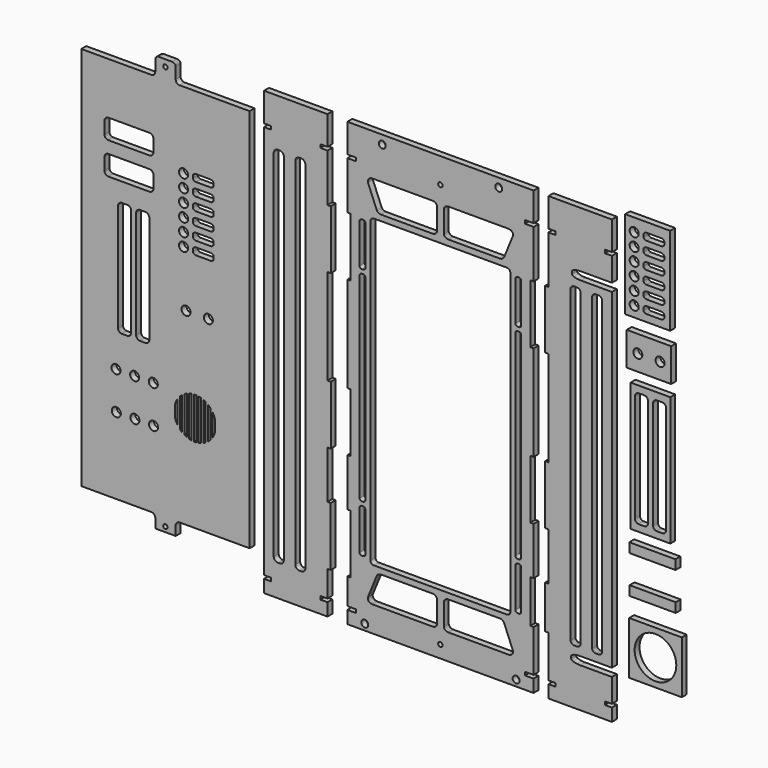
from build123d import *

# Parameters (mm, degrees)
F0_R     = 2.202959
F1_DEPTH = 3
F0_R_2   = 10.155753
F0_R_3   = 1.070008
F0_R_4   = 1.7


# Not quite as in the source:
# - ends of sketch curves that miss each other by under 0.0002 mm in the source are joined


with BuildPart() as f1:
    # F0 (on Front) → F1 (new body)
    with BuildSketch(Plane.XZ):
        Polygon((149.081306, 236.197677), (127.141025, 236.197677), (127.140998, 193.298079), (149.081279, 193.29808), align=None)
        with Locations((131.55197, 198.446738)):
            Circle(F0_R, mode=Mode.SUBTRACT)
        with Locations((131.55197, 204.737556)):
            Circle(F0_R, mode=Mode.SUBTRACT)
        with BuildLine():
            Line((136.085273, 197.958317), (136.085273, 198.935134))
            ThreePointArc((136.085273, 198.935134), (136.0896589586, 199.0280940094), (136.1030436281, 199.1201488772))
            ThreePointArc((136.1030436281, 199.1201488772), (136.1391328321, 199.2535893241), (136.193197735, 199.380812626))
            ThreePointArc((136.193197735, 199.380812626), (136.2769920688, 199.5198973917), (136.3792514469, 199.646028583))
            ThreePointArc((136.3792514469, 199.646028583), (136.5263451956, 199.7829173828), (136.6910356183, 199.8980356363))
            ThreePointArc((136.6910356183, 199.8980356363), (136.9043911921, 200.0070454279), (137.1306480519, 200.0858588099))
            ThreePointArc((137.1306480519, 200.0858588099), (137.3923568237, 200.1389087186), (137.6588280005, 200.1561971684))
            Line((137.6588280005, 200.1561971684), (144.671424, 200.156173))
            ThreePointArc((144.671424, 200.156173), (144.8570936657, 200.1479079079), (145.0412010492, 200.1224542646))
            ThreePointArc((145.0412010492, 200.1224542646), (145.2864322849, 200.0595456577), (145.5206188275, 199.963355651))
            ThreePointArc((145.5206188275, 199.963355651), (145.7043185156, 199.8563288234), (145.8714962897, 199.7249823204))
            ThreePointArc((145.8714962897, 199.7249823204), (145.9905352353, 199.6011912843), (146.0913932936, 199.4621871835))
            ThreePointArc((146.0913932936, 199.4621871835), (146.1594553593, 199.3336642686), (146.2089327204, 199.1969069205))
            ThreePointArc((146.2089327204, 199.1969069205), (146.2360068644, 199.0672875637), (146.2449620111, 198.935174))
            Line((146.2449620111, 198.935174), (146.244971, 197.958328))
            ThreePointArc((146.244971, 197.958328), (146.2405889845, 197.8654363974), (146.2272043351, 197.7733819345))
            ThreePointArc((146.2272043351, 197.7733819345), (146.1911151362, 197.6399415842), (146.137050265, 197.512718374))
            ThreePointArc((146.137050265, 197.512718374), (146.0532559312, 197.3736336083), (145.9509965531, 197.247502417))
            ThreePointArc((145.9509965531, 197.247502417), (145.8039024034, 197.1106141013), (145.6392121171, 196.9954958048))
            ThreePointArc((145.6392121171, 196.9954958048), (145.4258563643, 196.8864853826), (145.1995990175, 196.8076719359))
            ThreePointArc((145.1995990175, 196.8076719359), (144.9378906983, 196.7546222177), (144.6714199995, 196.7373338316))
            Line((144.6714199995, 196.7373338316), (137.65882, 196.737289))
            ThreePointArc((137.65882, 196.737289), (137.4731543343, 196.7456230921), (137.2890469508, 196.7710767354))
            ThreePointArc((137.2890469508, 196.7710767354), (137.0438156072, 196.8339850463), (136.8096289762, 196.9301749518))
            ThreePointArc((136.8096289762, 196.9301749518), (136.6259297618, 197.0372019881), (136.4587522077, 197.1685482297))
            ThreePointArc((136.4587522077, 197.1685482297), (136.3397129801, 197.2923394583), (136.2388547064, 197.4313438165))
            ThreePointArc((136.2388547064, 197.4313438165), (136.1707924688, 197.5598661194), (136.1213152796, 197.6966230795))
            ThreePointArc((136.1213152796, 197.6966230795), (136.0942411356, 197.8262424363), (136.085273, 197.958317))
        make_face(mode=Mode.SUBTRACT)
        with BuildLine():
            Line((136.085273, 204.249149), (136.085273, 205.225967))
            ThreePointArc((136.085273, 205.225967), (136.0896589586, 205.3188630094), (136.1030436281, 205.4109178772))
            ThreePointArc((136.1030436281, 205.4109178772), (136.1391328321, 205.5443583241), (136.193197735, 205.671581626))
            ThreePointArc((136.193197735, 205.671581626), (136.2769918588, 205.8106660924), (136.3792509481, 205.9367970484))
            ThreePointArc((136.3792509481, 205.9367970484), (136.5263449115, 206.0736861532), (136.6910356183, 206.1888046363))
            ThreePointArc((136.6910356183, 206.1888046363), (136.9043911921, 206.2978144279), (137.1306480519, 206.3766278099))
            ThreePointArc((137.1306480519, 206.3766278099), (137.3923568237, 206.4296777186), (137.6588280005, 206.4469661684))
            Line((137.6588280005, 206.4469661684), (144.671424, 206.446975))
            ThreePointArc((144.671424, 206.446975), (144.8570936657, 206.4386769079), (145.0412010492, 206.4132232646))
            ThreePointArc((145.0412010492, 206.4132232646), (145.2864322849, 206.3503146577), (145.5206188275, 206.254124651))
            ThreePointArc((145.5206188275, 206.254124651), (145.7043185156, 206.1470978234), (145.8714962897, 206.0157513204))
            ThreePointArc((145.8714962897, 206.0157513204), (145.9905352353, 205.8919602843), (146.0913932936, 205.7529561835))
            ThreePointArc((146.0913932936, 205.7529561835), (146.1594553593, 205.6244332686), (146.2089327204, 205.4876759205))
            ThreePointArc((146.2089327204, 205.4876759205), (146.2360068644, 205.3580565637), (146.2449620111, 205.225943))
            Line((146.2449620111, 205.225943), (146.244971, 204.24913))
            ThreePointArc((146.244971, 204.24913), (146.2405889845, 204.1562053974), (146.2272043351, 204.0641509345))
            ThreePointArc((146.2272043351, 204.0641509345), (146.1911151362, 203.9307105842), (146.137050265, 203.803487374))
            ThreePointArc((146.137050265, 203.803487374), (146.0532559312, 203.6644026083), (145.9509965531, 203.538271417))
            ThreePointArc((145.9509965531, 203.538271417), (145.8039024034, 203.4013831013), (145.6392121171, 203.2862648048))
            ThreePointArc((145.6392121171, 203.2862648048), (145.4258563643, 203.1772543826), (145.1995990175, 203.0984409359))
            ThreePointArc((145.1995990175, 203.0984409359), (144.9378906983, 203.0453912177), (144.6714199995, 203.0281028316))
            Line((144.6714199995, 203.0281028316), (137.65882, 203.028122))
            ThreePointArc((137.65882, 203.028122), (137.4731543343, 203.0363920921), (137.2890469508, 203.0618457354))
            ThreePointArc((137.2890469508, 203.0618457354), (137.0438156072, 203.1247540463), (136.8096289762, 203.2209439518))
            ThreePointArc((136.8096289762, 203.2209439518), (136.6259293014, 203.3279703009), (136.4587517103, 203.4593166796))
            ThreePointArc((136.4587517103, 203.4593166796), (136.3397129801, 203.5831084583), (136.2388547064, 203.7221128165))
            ThreePointArc((136.2388547064, 203.7221128165), (136.1707924688, 203.8506351194), (136.1213152796, 203.9873920795))
            ThreePointArc((136.1213152796, 203.9873920795), (136.0942411356, 204.1170114363), (136.085273, 204.249149))
        make_face(mode=Mode.SUBTRACT)
        with Locations((131.55197, 211.028375)):
            Circle(F0_R, mode=Mode.SUBTRACT)
        with Locations((131.55197, 217.319193)):
            Circle(F0_R, mode=Mode.SUBTRACT)
        with BuildLine():
            Line((136.085273, 210.539951), (136.085273, 211.516769))
            ThreePointArc((136.085273, 211.516769), (136.0896589586, 211.6096930094), (136.1030436281, 211.7017478772))
            ThreePointArc((136.1030436281, 211.7017478772), (136.1391326864, 211.835187903), (136.1931973308, 211.9624108317))
            ThreePointArc((136.1931973308, 211.9624108317), (136.2769920688, 212.1014953917), (136.3792514469, 212.227626583))
            ThreePointArc((136.3792514469, 212.227626583), (136.5263449115, 212.3645161532), (136.6910356183, 212.4796346363))
            ThreePointArc((136.6910356183, 212.4796346363), (136.90439155, 212.5886435808), (137.1306483061, 212.6674568793))
            ThreePointArc((137.1306483061, 212.6674568793), (137.3923568237, 212.7205077186), (137.6588280005, 212.7377961684))
            Line((137.6588280005, 212.7377961684), (144.671424, 212.737808))
            ThreePointArc((144.671424, 212.737808), (144.8570936657, 212.7295069079), (145.0412010492, 212.7040532646))
            ThreePointArc((145.0412010492, 212.7040532646), (145.2864322849, 212.6411446577), (145.5206188275, 212.544954651))
            ThreePointArc((145.5206188275, 212.544954651), (145.7043185156, 212.4379278234), (145.8714962897, 212.3065813204))
            ThreePointArc((145.8714962897, 212.3065813204), (145.9905352353, 212.1827902843), (146.0913932936, 212.0437861835))
            ThreePointArc((146.0913932936, 212.0437861835), (146.1594553593, 211.9152632686), (146.2089327204, 211.7785059205))
            ThreePointArc((146.2089327204, 211.7785059205), (146.2360068644, 211.6488865637), (146.2449620111, 211.516773))
            Line((146.2449620111, 211.516773), (146.244971, 210.539962))
            ThreePointArc((146.244971, 210.539962), (146.2405889845, 210.4470353974), (146.2272043351, 210.3549809345))
            ThreePointArc((146.2272043351, 210.3549809345), (146.1911154422, 210.2215404689), (146.1370506692, 210.0943171683))
            ThreePointArc((146.1370506692, 210.0943171683), (146.0532559312, 209.9552326083), (145.9509965531, 209.829101417))
            ThreePointArc((145.9509965531, 209.829101417), (145.8039024034, 209.6922131013), (145.6392121171, 209.5770948048))
            ThreePointArc((145.6392121171, 209.5770948048), (145.4258563643, 209.4680843826), (145.1995990175, 209.3892709359))
            ThreePointArc((145.1995990175, 209.3892709359), (144.9378906983, 209.3362212177), (144.6714199995, 209.3189328316))
            Line((144.6714199995, 209.3189328316), (137.65882, 209.318954))
            ThreePointArc((137.65882, 209.318954), (137.4731543343, 209.3272220921), (137.2890469508, 209.3526757354))
            ThreePointArc((137.2890469508, 209.3526757354), (137.0438156072, 209.4155840463), (136.8096289762, 209.5117739518))
            ThreePointArc((136.8096289762, 209.5117739518), (136.6259293014, 209.6188003009), (136.4587517103, 209.7501466796))
            ThreePointArc((136.4587517103, 209.7501466796), (136.3397132522, 209.8739381332), (136.2388551559, 210.0129420974))
            ThreePointArc((136.2388551559, 210.0129420974), (136.1707926407, 210.1414647314), (136.1213152796, 210.2782220795))
            ThreePointArc((136.1213152796, 210.2782220795), (136.0942411356, 210.4078414363), (136.085273, 210.539951))
        make_face(mode=Mode.SUBTRACT)
        with BuildLine():
            Line((136.085273, 216.830784), (136.085273, 217.807602))
            ThreePointArc((136.085273, 217.807602), (136.0896589586, 217.9005230094), (136.1030436281, 217.9925778772))
            ThreePointArc((136.1030436281, 217.9925778772), (136.1391326864, 218.126017903), (136.1931973308, 218.2532408317))
            ThreePointArc((136.1931973308, 218.2532408317), (136.2769920688, 218.3923253917), (136.3792514469, 218.518456583))
            ThreePointArc((136.3792514469, 218.518456583), (136.5263449115, 218.6553461532), (136.6910356183, 218.7704646363))
            ThreePointArc((136.6910356183, 218.7704646363), (136.9043914289, 218.8794735291), (137.1306480519, 218.9582868099))
            ThreePointArc((137.1306480519, 218.9582868099), (137.3923568223, 219.0113367184), (137.6588279977, 219.0286251684))
            Line((137.6588279977, 219.0286251684), (144.671424, 219.02861))
            ThreePointArc((144.671424, 219.02861), (144.8570936657, 219.0203369079), (145.0412010492, 218.9948832646))
            ThreePointArc((145.0412010492, 218.9948832646), (145.2864324952, 218.9319745879), (145.5206192247, 218.8357844547))
            ThreePointArc((145.5206192247, 218.8357844547), (145.7043186986, 218.7287576991), (145.8714962897, 218.5974113204))
            ThreePointArc((145.8714962897, 218.5974113204), (145.9905352353, 218.4736202843), (146.0913932936, 218.3346161835))
            ThreePointArc((146.0913932936, 218.3346161835), (146.1594553593, 218.2060932686), (146.2089327204, 218.0693359205))
            ThreePointArc((146.2089327204, 218.0693359205), (146.2360068644, 217.9397165637), (146.2449620111, 217.807603))
            Line((146.2449620111, 217.807603), (146.244971, 216.830764))
            ThreePointArc((146.244971, 216.830764), (146.2405889376, 216.7378649089), (146.2272041468, 216.6458099713))
            ThreePointArc((146.2272041468, 216.6458099713), (146.1911152819, 216.5123700053), (146.1370506692, 216.3851471683))
            ThreePointArc((146.1370506692, 216.3851471683), (146.0532559312, 216.2460626083), (145.9509965531, 216.119931417))
            ThreePointArc((145.9509965531, 216.119931417), (145.8039022033, 215.9830429396), (145.6392116759, 215.8679245402))
            ThreePointArc((145.6392116759, 215.8679245402), (145.4258561276, 215.7589142814), (145.1995990175, 215.6801009359))
            ThreePointArc((145.1995990175, 215.6801009359), (144.9378906983, 215.6270512177), (144.6714199995, 215.6097628316))
            Line((144.6714199995, 215.6097628316), (137.65882, 215.609756))
            ThreePointArc((137.65882, 215.609756), (137.4731544253, 215.6180520837), (137.2890471305, 215.643505702))
            ThreePointArc((137.2890471305, 215.643505702), (137.043815693, 215.7064140178), (136.8096289762, 215.8026039518))
            ThreePointArc((136.8096289762, 215.8026039518), (136.6259293014, 215.9096303009), (136.4587517103, 216.0409766796))
            ThreePointArc((136.4587517103, 216.0409766796), (136.3397127647, 216.1647677157), (136.2388547064, 216.3037718165))
            ThreePointArc((136.2388547064, 216.3037718165), (136.1707926407, 216.4322947314), (136.1213152796, 216.5690520795))
            ThreePointArc((136.1213152796, 216.5690520795), (136.0942411356, 216.6986714363), (136.085273, 216.830784))
        make_face(mode=Mode.SUBTRACT)
        with Locations((131.55197, 223.610012)):
            Circle(F0_R, mode=Mode.SUBTRACT)
        with Locations((131.55197, 229.90083)):
            Circle(F0_R, mode=Mode.SUBTRACT)
        with BuildLine():
            Line((136.085273, 223.121586), (136.085273, 224.098404))
            ThreePointArc((136.085273, 224.098404), (136.0896589586, 224.1913530094), (136.1030436281, 224.2834078772))
            ThreePointArc((136.1030436281, 224.2834078772), (136.1391326864, 224.416847903), (136.1931973308, 224.5440708317))
            ThreePointArc((136.1931973308, 224.5440708317), (136.2769920688, 224.6831553917), (136.3792514469, 224.809286583))
            ThreePointArc((136.3792514469, 224.809286583), (136.5263453957, 224.9461755445), (136.6910360594, 225.061293901))
            ThreePointArc((136.6910360594, 225.061293901), (136.9043914289, 225.1703035291), (137.1306480519, 225.2491168099))
            ThreePointArc((137.1306480519, 225.2491168099), (137.3923568237, 225.3021667186), (137.6588280005, 225.3194551684))
            Line((137.6588280005, 225.3194551684), (144.671424, 225.319442))
            ThreePointArc((144.671424, 225.319442), (144.8570936648, 225.311166908), (145.0412010492, 225.2857132646))
            ThreePointArc((145.0412010492, 225.2857132646), (145.2864324952, 225.2228045879), (145.5206192247, 225.1266144547))
            ThreePointArc((145.5206192247, 225.1266144547), (145.7043186986, 225.0195876991), (145.8714962897, 224.8882413204))
            ThreePointArc((145.8714962897, 224.8882413204), (145.9905352353, 224.7644502843), (146.0913932936, 224.6254461835))
            ThreePointArc((146.0913932936, 224.6254461835), (146.1594553593, 224.4969232686), (146.2089327204, 224.3601659205))
            ThreePointArc((146.2089327204, 224.3601659205), (146.2360068644, 224.2305465637), (146.2449620111, 224.098433))
            Line((146.2449620111, 224.098433), (146.244971, 223.121597))
            ThreePointArc((146.244971, 223.121597), (146.2405889376, 223.0286949089), (146.2272041468, 222.9366399713))
            ThreePointArc((146.2272041468, 222.9366399713), (146.1911152819, 222.8032000053), (146.1370506692, 222.6759771683))
            ThreePointArc((146.1370506692, 222.6759771683), (146.0532559312, 222.5368926083), (145.9509965531, 222.410761417))
            ThreePointArc((145.9509965531, 222.410761417), (145.8039022033, 222.2738729396), (145.6392116759, 222.1587545402))
            ThreePointArc((145.6392116759, 222.1587545402), (145.4258561276, 222.0497442814), (145.1995990175, 221.9709309359))
            ThreePointArc((145.1995990175, 221.9709309359), (144.9378906983, 221.9178812177), (144.6714199995, 221.9005928316))
            Line((144.6714199995, 221.9005928316), (137.65882, 221.900589))
            ThreePointArc((137.65882, 221.900589), (137.4731544253, 221.9088820837), (137.2890471305, 221.934335702))
            ThreePointArc((137.2890471305, 221.934335702), (137.043815693, 221.9972440178), (136.8096289762, 222.0934339518))
            ThreePointArc((136.8096289762, 222.0934339518), (136.6259293014, 222.2004603009), (136.4587517103, 222.3318066796))
            ThreePointArc((136.4587517103, 222.3318066796), (136.3397127647, 222.4555977157), (136.2388547064, 222.5946018165))
            ThreePointArc((136.2388547064, 222.5946018165), (136.1707926407, 222.7231247314), (136.1213152796, 222.8598820795))
            ThreePointArc((136.1213152796, 222.8598820795), (136.0942411356, 222.9895014363), (136.085273, 223.121586))
        make_face(mode=Mode.SUBTRACT)
        with BuildLine():
            Line((136.085273, 229.412418), (136.085273, 230.389236))
            ThreePointArc((136.085273, 230.389236), (136.0896590532, 230.4821219956), (136.1030438164, 230.5741768404))
            ThreePointArc((136.1030438164, 230.5741768404), (136.1391326864, 230.707616903), (136.1931973308, 230.8348398317))
            ThreePointArc((136.1931973308, 230.8348398317), (136.2769920688, 230.9739243917), (136.3792514469, 231.100055583))
            ThreePointArc((136.3792514469, 231.100055583), (136.5263453957, 231.2369445445), (136.6910360594, 231.352062901))
            ThreePointArc((136.6910360594, 231.352062901), (136.9043914289, 231.4610725291), (137.1306480519, 231.5398858099))
            ThreePointArc((137.1306480519, 231.5398858099), (137.3923568237, 231.5929357186), (137.6588280005, 231.6102241684))
            Line((137.6588280005, 231.6102241684), (144.671424, 231.610244))
            ThreePointArc((144.671424, 231.610244), (144.8570935747, 231.6019349163), (145.0412008695, 231.576481298))
            ThreePointArc((145.0412008695, 231.576481298), (145.2864324952, 231.5135735879), (145.5206192247, 231.4173834547))
            ThreePointArc((145.5206192247, 231.4173834547), (145.7043186986, 231.3103566991), (145.8714962897, 231.1790103204))
            ThreePointArc((145.8714962897, 231.1790103204), (145.9905352353, 231.0552192843), (146.0913932936, 230.9162151835))
            ThreePointArc((146.0913932936, 230.9162151835), (146.1594553593, 230.7876922686), (146.2089327204, 230.6509349205))
            ThreePointArc((146.2089327204, 230.6509349205), (146.2360068644, 230.5213155637), (146.2449620111, 230.389202))
            Line((146.2449620111, 230.389202), (146.244971, 229.412399))
            ThreePointArc((146.244971, 229.412399), (146.2405890323, 229.3194638951), (146.2272043351, 229.2274089345))
            ThreePointArc((146.2272043351, 229.2274089345), (146.1911152819, 229.0939690053), (146.1370506692, 228.9667461683))
            ThreePointArc((146.1370506692, 228.9667461683), (146.0532559312, 228.8276616083), (145.9509965531, 228.701530417))
            ThreePointArc((145.9509965531, 228.701530417), (145.8039022033, 228.5646419396), (145.6392116759, 228.4495235402))
            ThreePointArc((145.6392116759, 228.4495235402), (145.4258561276, 228.3405132814), (145.1995990175, 228.2616999359))
            ThreePointArc((145.1995990175, 228.2616999359), (144.9378906983, 228.2086502177), (144.6714199995, 228.1913618316))
            Line((144.6714199995, 228.1913618316), (137.65882, 228.191391))
            ThreePointArc((137.65882, 228.191391), (137.4731544253, 228.1996510837), (137.2890471305, 228.225104702))
            ThreePointArc((137.2890471305, 228.225104702), (137.043815397, 228.2880121161), (136.8096285789, 228.3842021481))
            ThreePointArc((136.8096285789, 228.3842021481), (136.6259293014, 228.4912293009), (136.4587517103, 228.6225756796))
            ThreePointArc((136.4587517103, 228.6225756796), (136.3397127647, 228.7463667157), (136.2388547064, 228.8853708165))
            ThreePointArc((136.2388547064, 228.8853708165), (136.1707926407, 229.0138937314), (136.1213152796, 229.1506510795))
            ThreePointArc((136.1213152796, 229.1506510795), (136.0942411356, 229.2802704363), (136.085273, 229.412418))
        make_face(mode=Mode.SUBTRACT)
    extrude(amount=F1_DEPTH)


with BuildPart() as f1b:
    # F0 (on Front) → F1, piece 2 (new body)
    with BuildSketch(Plane.XZ):
        Polygon((149.531287, 186.842239), (127.908335, 186.842239), (127.908332, 170.604296), (149.531285, 170.604293), align=None)
        with Locations((133.322705, 178.423265)):
            Circle(F0_R, mode=Mode.SUBTRACT)
        with Locations((144.172127, 178.423265)):
            Circle(F0_R, mode=Mode.SUBTRACT)
    extrude(amount=F1_DEPTH)


with BuildPart() as f1c:
    # F0 (on Front) → F1, piece 3 (new body)
    with BuildSketch(Plane.XZ):
        Polygon((149.148414, 102.077835), (149.148414, 164.846023), (129.805164, 164.846023), (129.805152, 102.077835), align=None)
        with BuildLine():
            Line((131.877479, 107.362741), (131.877479, 159.561111))
            ThreePointArc((131.877479, 159.561111), (131.8860753429, 159.7528666826), (131.9124345455, 159.9430098984))
            ThreePointArc((131.9124345455, 159.9430098984), (131.9817521094, 160.2112770565), (132.0870892741, 160.4675508647))
            ThreePointArc((132.0870892741, 160.4675508647), (132.2224535312, 160.7004077271), (132.3880909612, 160.9127990348))
            ThreePointArc((132.3880909612, 160.9127990348), (132.5784574622, 161.097850966), (132.7925955322, 161.2547857412))
            ThreePointArc((132.7925955322, 161.2547857412), (133.0182389657, 161.3758644274), (133.2586187772, 161.4641397701))
            ThreePointArc((133.2586187772, 161.4641397701), (133.5059624267, 161.516856919), (133.758261999, 161.5342604355))
            Line((133.758261999, 161.5342604355), (136.444434, 161.534256))
            ThreePointArc((136.444434, 161.534256), (136.617410764, 161.5261728569), (136.7888031406, 161.5015097269))
            ThreePointArc((136.7888031406, 161.5015097269), (137.0280071338, 161.4376722199), (137.2562208659, 161.3416917339))
            ThreePointArc((137.2562208659, 161.3416917339), (137.4838475209, 161.2058789815), (137.6901506087, 161.0394516544))
            ThreePointArc((137.6901506087, 161.0394516544), (137.8732727738, 160.8442350414), (138.0281907358, 160.6259608383))
            ThreePointArc((138.0281907358, 160.6259608383), (138.1549407287, 160.3830612142), (138.2475006936, 160.1251881968))
            ThreePointArc((138.2475006936, 160.1251881968), (138.3059907507, 159.8458472937), (138.3252329197, 159.5610979982))
            Line((138.3252329197, 159.5610979982), (138.325233, 107.362747))
            ThreePointArc((138.325233, 107.362747), (138.3166286571, 107.1709513174), (138.2902694545, 106.9808081016))
            ThreePointArc((138.2902694545, 106.9808081016), (138.2209518906, 106.7125409435), (138.1156147259, 106.4562671353))
            ThreePointArc((138.1156147259, 106.4562671353), (137.9802499882, 106.2234110412), (137.8146129807, 106.0110200173))
            ThreePointArc((137.8146129807, 106.0110200173), (137.6242463998, 105.8259677628), (137.4101081829, 105.6690327102))
            ThreePointArc((137.4101081829, 105.6690327102), (137.1844646642, 105.5479544063), (136.9440849558, 105.4596791526))
            ThreePointArc((136.9440849558, 105.4596791526), (136.6967415733, 105.406961081), (136.444442001, 105.3895575645))
            Line((136.444442001, 105.3895575645), (133.758277, 105.389572))
            ThreePointArc((133.758277, 105.389572), (133.585293236, 105.3976451431), (133.4139008594, 105.4223082731))
            ThreePointArc((133.4139008594, 105.4223082731), (133.1746966533, 105.4861458529), (132.9464827322, 105.5821264686))
            ThreePointArc((132.9464827322, 105.5821264686), (132.7188567585, 105.7179398239), (132.51255389, 105.8843668817))
            ThreePointArc((132.51255389, 105.8843668817), (132.3294306231, 106.0795824731), (132.1745125366, 106.2978567164))
            ThreePointArc((132.1745125366, 106.2978567164), (132.0477632713, 106.5407567858), (131.9552033064, 106.7986298032))
            ThreePointArc((131.9552033064, 106.7986298032), (131.8967132493, 107.0779707063), (131.877479, 107.362741))
        make_face(mode=Mode.SUBTRACT)
        with BuildLine():
            Line((140.688087, 107.207711), (140.688087, 159.406082))
            ThreePointArc((140.688087, 159.406082), (140.6967032609, 159.5978447864), (140.723062399, 159.787988112))
            ThreePointArc((140.723062399, 159.787988112), (140.7923803499, 160.0562557788), (140.8977178669, 160.3125300657))
            ThreePointArc((140.8977178669, 160.3125300657), (141.0330827823, 160.5453860985), (141.1987199612, 160.7577770348))
            ThreePointArc((141.1987199612, 160.7577770348), (141.3890864622, 160.942828966), (141.6032245322, 161.0997637412))
            ThreePointArc((141.6032245322, 161.0997637412), (141.8288679163, 161.2208428545), (142.0692479669, 161.3091181144))
            ThreePointArc((142.0692479669, 161.3091181144), (142.3165914276, 161.3618359191), (142.5688910007, 161.3792394355))
            Line((142.5688910007, 161.3792394355), (145.255042, 161.379257))
            ThreePointArc((145.255042, 161.379257), (145.4280241718, 161.3711509132), (145.5994169542, 161.346487763))
            ThreePointArc((145.5994169542, 161.346487763), (145.8386209304, 161.2826499475), (146.0668346634, 161.186669332))
            ThreePointArc((146.0668346634, 161.186669332), (146.2944611876, 161.0508565172), (146.5007641448, 160.8844291557))
            ThreePointArc((146.5007641448, 160.8844291557), (146.6838872593, 160.6892134476), (146.838805181, 160.4709391108))
            ThreePointArc((146.838805181, 160.4709391108), (146.9655538882, 160.2280388501), (147.0581137681, 159.9701659342))
            ThreePointArc((147.0581137681, 159.9701659342), (147.1166037692, 159.6908251598), (147.1358459197, 159.4060760002))
            Line((147.1358459197, 159.4060760002), (147.135841, 107.207718))
            ThreePointArc((147.135841, 107.207718), (147.1272426487, 107.0159602262), (147.1008834209, 106.8258169216))
            ThreePointArc((147.1008834209, 106.8258169216), (147.0315657917, 106.5575496465), (146.92622853, 106.3012757384))
            ThreePointArc((146.92622853, 106.3012757384), (146.7908636556, 106.0684195492), (146.6252264838, 105.8560284622))
            ThreePointArc((146.6252264838, 105.8560284622), (146.4348601153, 105.6709765223), (146.2207221829, 105.5140417102))
            ThreePointArc((146.2207221829, 105.5140417102), (145.9950790343, 105.3929625726), (145.7546992228, 105.3046872299))
            ThreePointArc((145.7546992228, 105.3046872299), (145.5073550491, 105.2519701478), (145.255055001, 105.2345665645))
            Line((145.255055001, 105.2345665645), (142.568885, 105.234542))
            ThreePointArc((142.568885, 105.234542), (142.395922236, 105.2426541431), (142.2245298594, 105.2673172731))
            ThreePointArc((142.2245298594, 105.2673172731), (141.9853258662, 105.3311547801), (141.7571121341, 105.4271352661))
            ThreePointArc((141.7571121341, 105.4271352661), (141.5294851787, 105.5629482277), (141.3231818552, 105.7293758443))
            ThreePointArc((141.3231818552, 105.7293758443), (141.1400592262, 105.9245919586), (140.9851412642, 106.1428661617))
            ThreePointArc((140.9851412642, 106.1428661617), (140.8583921666, 106.3857660249), (140.7658323064, 106.6436388032))
            ThreePointArc((140.7658323064, 106.6436388032), (140.7073422494, 106.9229797053), (140.688087, 107.207711))
        make_face(mode=Mode.SUBTRACT)
    extrude(amount=F1_DEPTH)


with BuildPart() as f1d:
    # F0 (on Front) → F1, piece 4 (new body)
    with BuildSketch(Plane.XZ):
        Polygon((151.646735, 96.16658), (129.152748, 96.16658), (129.152747, 91.539375), (151.646735, 91.539352), align=None)
    extrude(amount=F1_DEPTH)


with BuildPart() as f1e:
    # F0 (on Front) → F1, piece 5 (new body)
    with BuildSketch(Plane.XZ):
        Polygon((151.78849, 77.786972), (129.294502, 77.786972), (129.294501, 73.159767), (151.788489, 73.159774), align=None)
    extrude(amount=F1_DEPTH)


with BuildPart() as f1f:
    # F0 (on Front) → F1, piece 6 (new body)
    with BuildSketch(Plane.XZ):
        Polygon((154.731391, 63.657974), (129.065035, 63.657974), (129.06504, 37.991548), (154.731396, 37.991531), align=None)
        with Locations((141.898244, 50.824752)):
            Circle(F0_R_2, mode=Mode.SUBTRACT)
    extrude(amount=F1_DEPTH)


with BuildPart() as f1g:
    # F0 (on Front) → F1, piece 7 (new body)
    with BuildSketch(Plane.XZ):
        with BuildLine():
            Line((-101.744496, 26.968313), (-91.797555, 26.968307))
            Line((-91.797555, 26.968307), (-91.797555, 31.523385))
            ThreePointArc((-91.797555, 31.523385), (-91.2444973796, 32.8585853796), (-89.909303, 33.411641))
            Line((-89.909303, 33.411641), (-55.766574, 33.411636))
            Line((-55.766574, 33.411636), (-55.766579, 220.892908))
            Line((-55.766579, 220.892908), (-89.909308, 220.892898))
            ThreePointArc((-89.909308, 220.892898), (-91.2444973796, 221.4459786204), (-91.797553, 222.781173))
            Line((-91.797553, 222.781173), (-91.797555, 228.378916))
            ThreePointArc((-91.797555, 228.378916), (-91.8083202781, 228.531234944), (-91.8407919733, 228.6804330079))
            ThreePointArc((-91.8407919733, 228.6804330079), (-91.900318253, 228.8383062542), (-91.9818391269, 228.9860279176))
            ThreePointArc((-91.9818391269, 228.9860279176), (-92.1032384979, 229.1465808235), (-92.2457160659, 229.2887609241))
            ThreePointArc((-92.2457160659, 229.2887609241), (-92.4468746466, 229.4404245888), (-92.6667687793, 229.5633604667))
            ThreePointArc((-92.6667687793, 229.5633604667), (-92.9576892393, 229.6772708933), (-93.2615219353, 229.750044386))
            ThreePointArc((-93.2615219353, 229.750044386), (-93.4729111165, 229.7767891473), (-93.6858069985, 229.7855070346))
            Line((-93.6858069985, 229.7855070346), (-99.856246, 229.785476))
            ThreePointArc((-99.856246, 229.785476), (-100.1948080556, 229.7631344676), (-100.52705285, 229.694329465))
            ThreePointArc((-100.52705285, 229.694329465), (-100.8030563465, 229.596267756), (-101.0628299668, 229.4609469458))
            ThreePointArc((-101.0628299668, 229.4609469458), (-101.2544138967, 229.3243281971), (-101.4249500251, 229.1621970229))
            ThreePointArc((-101.4249500251, 229.1621970229), (-101.5371901885, 229.0205417438), (-101.6290080057, 228.864870502))
            ThreePointArc((-101.6290080057, 228.864870502), (-101.6898088561, 228.7170859721), (-101.728832691, 228.5621209454))
            ThreePointArc((-101.728832691, 228.5621209454), (-101.7406552447, 228.4708635824), (-101.7445014685, 228.3789240009))
            Line((-101.7445014685, 228.3789240009), (-101.744496, 222.781148))
            ThreePointArc((-101.744496, 222.781148), (-102.2975506204, 221.4459786204), (-103.632745, 220.892923))
            Line((-103.632745, 220.892923), (-137.775473, 220.892898))
            Line((-137.775473, 220.892898), (-137.775473, 33.411626))
            Line((-137.775473, 33.411626), (-103.632745, 33.411636))
            ThreePointArc((-103.632745, 33.411636), (-102.2975506204, 32.8585853796), (-101.744495, 31.523391))
            Line((-101.744495, 31.523391), (-101.744496, 26.968313))
        make_face()
        with Locations((-96.801736, 29.378372)):
            Circle(F0_R_3, mode=Mode.SUBTRACT)
        with Locations((-120.72239, 70.697708)):
            Circle(F0_R, mode=Mode.SUBTRACT)
        with Locations((-111.645768, 70.697708)):
            Circle(F0_R, mode=Mode.SUBTRACT)
        with Locations((-102.569146, 70.697708)):
            Circle(F0_R, mode=Mode.SUBTRACT)
        with Locations((-120.864133, 89.077316)):
            Circle(F0_R, mode=Mode.SUBTRACT)
        with Locations((-111.787511, 89.077316)):
            Circle(F0_R, mode=Mode.SUBTRACT)
        with Locations((-102.710889, 89.077316)):
            Circle(F0_R, mode=Mode.SUBTRACT)
        with BuildLine():
            Line((-90.944497, 85.980503), (-90.944497, 74.971939))
            ThreePointArc((-90.944497, 74.971939), (-91.6096041163, 76.1748582778), (-92.1061815482, 77.4565841407))
            Line((-92.1061815482, 77.4565841407), (-92.106179, 83.495834))
            ThreePointArc((-92.106179, 83.495834), (-91.6096041163, 84.7775637222), (-90.944497, 85.980503))
        make_face(mode=Mode.SUBTRACT)
        with BuildLine():
            Line((-88.649857, 88.488728), (-88.649857, 72.463729))
            ThreePointArc((-88.649857, 72.463729), (-89.2512179138, 72.9706555827), (-89.8115439637, 73.5226170341))
            Line((-89.8115439637, 73.5226170341), (-89.811547, 87.429824))
            ThreePointArc((-89.811547, 87.429824), (-89.2512179138, 87.9817664173), (-88.649857, 88.488728))
        make_face(mode=Mode.SUBTRACT)
        with BuildLine():
            Line((-86.355218, 89.834239), (-86.355218, 71.118209))
            ThreePointArc((-86.355218, 71.118209), (-86.945338716, 71.3895409514), (-87.5169066697, 71.6980525677))
            Line((-87.5169066697, 71.6980525677), (-87.516908, 89.254379))
            ThreePointArc((-87.516908, 89.254379), (-86.945338716, 89.5628810486), (-86.355218, 89.834239))
        make_face(mode=Mode.SUBTRACT)
        with BuildLine():
            Line((-84.060578, 90.496909), (-84.060578, 70.455551))
            ThreePointArc((-84.060578, 70.455551), (-84.6452713128, 70.5695630283), (-85.2222689533, 70.717679162))
            Line((-85.2222689533, 70.717679162), (-85.222268, 90.234756))
            ThreePointArc((-85.222268, 90.234756), (-84.6452713128, 90.3828589717), (-84.060578, 90.496909))
        make_face(mode=Mode.SUBTRACT)
        with BuildLine():
            ThreePointArc((-81.7659440471, 70.3408837412), (-82.3466848203, 70.3206536887), (-82.9276319979, 70.3336720418))
            Line((-82.9276319979, 70.3336720418), (-82.927628, 90.618759))
            ThreePointArc((-82.927628, 90.618759), (-82.3466847948, 90.6317683111), (-81.7659440471, 90.6115382588))
            Line((-81.7659440471, 90.6115382588), (-81.7659440471, 70.3408837412))
        make_face(mode=Mode.SUBTRACT)
        with BuildLine():
            ThreePointArc((-79.4713070929, 70.7548433073), (-80.0480636184, 70.5988707255), (-80.6329941083, 70.4770846097))
            Line((-80.6329941083, 70.4770846097), (-80.632996, 90.475357))
            ThreePointArc((-80.632996, 90.475357), (-80.0480636184, 90.3535512745), (-79.4713070929, 90.1975786927))
            Line((-79.4713070929, 90.1975786927), (-79.4713070929, 70.7548433073))
        make_face(mode=Mode.SUBTRACT)
        with BuildLine():
            ThreePointArc((-77.1766694955, 71.7725108241), (-77.7478428847, 71.4536765711), (-78.3383570554, 71.1722741267))
            Line((-78.3383570554, 71.1722741267), (-78.338357, 89.780166))
            ThreePointArc((-78.338357, 89.780166), (-77.7478428847, 89.4987454289), (-77.1766694955, 89.1799111759))
            Line((-77.1766694955, 89.1799111759), (-77.1766694955, 71.7725108241))
        make_face(mode=Mode.SUBTRACT)
        with BuildLine():
            ThreePointArc((-74.8820325842, 73.659093529), (-75.4413056554, 73.0883573773), (-76.0437196066, 72.563358754))
            Line((-76.0437196066, 72.563358754), (-76.043717, 88.389083))
            ThreePointArc((-76.043717, 88.389083), (-75.4413056554, 87.8640646227), (-74.8820325842, 87.293328471))
            Line((-74.8820325842, 87.293328471), (-74.8820325842, 73.659093529))
        make_face(mode=Mode.SUBTRACT)
        with BuildLine():
            ThreePointArc((-72.5873950471, 77.8953090124), (-73.068478001, 76.4911978146), (-73.7490822371, 75.1722031452))
            Line((-73.7490822371, 75.1722031452), (-73.749078, 85.780227))
            ThreePointArc((-73.749078, 85.780227), (-73.068478358, 84.4612250224), (-72.5873952929, 83.057113923))
            Line((-72.5873952929, 83.057113923), (-72.5873950471, 77.8953090124))
        make_face(mode=Mode.SUBTRACT)
        with Locations((-86.736985, 125.223404)):
            Circle(F0_R, mode=Mode.SUBTRACT)
        with Locations((-75.887559, 125.223404)):
            Circle(F0_R, mode=Mode.SUBTRACT)
        with BuildLine():
            Line((-111.094258, 106.968576), (-111.094258, 159.166946))
            ThreePointArc((-111.094258, 159.166946), (-111.0856556487, 159.3587267738), (-111.0592964209, 159.5488700784))
            ThreePointArc((-111.0592964209, 159.5488700784), (-110.9899787917, 159.8171373535), (-110.88464153, 160.0734112616))
            ThreePointArc((-110.88464153, 160.0734112616), (-110.7492764688, 160.3062677271), (-110.5836390388, 160.5186590348))
            ThreePointArc((-110.5836390388, 160.5186590348), (-110.3932725378, 160.703710966), (-110.1791344678, 160.8606457412))
            ThreePointArc((-110.1791344678, 160.8606457412), (-109.9534916486, 160.9817246007), (-109.7131122228, 161.0699997701))
            ThreePointArc((-109.7131122228, 161.0699997701), (-109.4657680491, 161.1227168522), (-109.213468001, 161.1401204355))
            Line((-109.213468001, 161.1401204355), (-106.527299, 161.140121))
            ThreePointArc((-106.527299, 161.140121), (-106.3543352224, 161.1320329507), (-106.1829428234, 161.1073699133))
            ThreePointArc((-106.1829428234, 161.1073699133), (-105.9437388662, 161.0435322199), (-105.7155251341, 160.9475517339))
            ThreePointArc((-105.7155251341, 160.9475517339), (-105.4878981787, 160.8117387723), (-105.2815948552, 160.6453111557))
            ThreePointArc((-105.2815948552, 160.6453111557), (-105.0984722262, 160.4500950414), (-104.9435542642, 160.2318208383))
            ThreePointArc((-104.9435542642, 160.2318208383), (-104.8168051118, 159.9889208501), (-104.7242452319, 159.7310479342))
            ThreePointArc((-104.7242452319, 159.7310479342), (-104.6657552308, 159.4517071598), (-104.6465130803, 159.1669580002))
            Line((-104.6465130803, 159.1669580002), (-104.646508, 106.968582))
            ThreePointArc((-104.646508, 106.968582), (-104.6551163513, 106.7768112262), (-104.6814755791, 106.5866679216))
            ThreePointArc((-104.6814755791, 106.5866679216), (-104.7507932083, 106.3184006465), (-104.85613047, 106.0621267384))
            ThreePointArc((-104.85613047, 106.0621267384), (-104.9914951358, 105.8292708578), (-105.1571320193, 105.6168800173))
            ThreePointArc((-105.1571320193, 105.6168800173), (-105.3474986002, 105.4318277628), (-105.5616368171, 105.2748927102))
            ThreePointArc((-105.5616368171, 105.2748927102), (-105.7872803358, 105.1538144063), (-106.0276600442, 105.0655391526))
            ThreePointArc((-106.0276600442, 105.0655391526), (-106.2750039509, 105.0128211478), (-106.527303999, 104.9954175645))
            Line((-106.527303999, 104.9954175645), (-109.213467, 104.995407))
            ThreePointArc((-109.213467, 104.995407), (-109.386436764, 105.0035051431), (-109.5578291406, 105.0281682731))
            ThreePointArc((-109.5578291406, 105.0281682731), (-109.7970333467, 105.0920058529), (-110.0252472678, 105.1879864686))
            ThreePointArc((-110.0252472678, 105.1879864686), (-110.2528735419, 105.3238000331), (-110.4591766461, 105.4902273804))
            ThreePointArc((-110.4591766461, 105.4902273804), (-110.6422997738, 105.6854429586), (-110.7972177358, 105.9037171617))
            ThreePointArc((-110.7972177358, 105.9037171617), (-110.9239668334, 106.1466170249), (-111.0165266936, 106.4044898032))
            ThreePointArc((-111.0165266936, 106.4044898032), (-111.0750167506, 106.6838307053), (-111.094258, 106.968576))
        make_face(mode=Mode.SUBTRACT)
        with BuildLine():
            Line((-119.904877, 107.123605), (-119.904877, 159.321975))
            ThreePointArc((-119.904877, 159.321975), (-119.8962687475, 159.5137476952), (-119.8699096345, 159.7038909319))
            ThreePointArc((-119.8699096345, 159.7038909319), (-119.8005920459, 159.9721585902), (-119.6952547259, 160.2284328647))
            ThreePointArc((-119.6952547259, 160.2284328647), (-119.5598895285, 160.4612886388), (-119.3942524838, 160.6736795378))
            ThreePointArc((-119.3942524838, 160.6736795378), (-119.2038859115, 160.85873165), (-118.9897477316, 161.0156665747))
            ThreePointArc((-118.9897477316, 161.0156665747), (-118.7641046642, 161.1367455937), (-118.5237249558, 161.2250208474))
            ThreePointArc((-118.5237249558, 161.2250208474), (-118.2763810781, 161.2777389885), (-118.024081001, 161.2951424338))
            Line((-118.024081001, 161.2951424338), (-115.337918, 161.29512))
            ThreePointArc((-115.337918, 161.29512), (-115.1649488275, 161.2870539132), (-114.9935560458, 161.262390763))
            ThreePointArc((-114.9935560458, 161.262390763), (-114.7543516533, 161.1985541471), (-114.5261377322, 161.1025735314))
            ThreePointArc((-114.5261377322, 161.1025735314), (-114.2985117585, 160.9667601761), (-114.09220889, 160.8003331183))
            ThreePointArc((-114.09220889, 160.8003331183), (-113.9090862262, 160.6051170414), (-113.7541682642, 160.3868428383))
            ThreePointArc((-113.7541682642, 160.3868428383), (-113.6274186353, 160.1439430455), (-113.534858569, 159.8860701223))
            ThreePointArc((-113.534858569, 159.8860701223), (-113.476368181, 159.6067287984), (-113.4571260823, 159.3219789982))
            Line((-113.4571260823, 159.3219789982), (-113.457127, 107.123611))
            ThreePointArc((-113.457127, 107.123611), (-113.4657302525, 106.9318333048), (-113.4920893655, 106.7416900681))
            ThreePointArc((-113.4920893655, 106.7416900681), (-113.5614072511, 106.4734225181), (-113.666744671, 106.2171483312))
            ThreePointArc((-113.666744671, 106.2171483312), (-113.8021094715, 105.9842923612), (-113.9677465162, 105.7719014622))
            ThreePointArc((-113.9677465162, 105.7719014622), (-114.1581128847, 105.5868495223), (-114.3722508171, 105.4299147102))
            ThreePointArc((-114.3722508171, 105.4299147102), (-114.5978940924, 105.3088355156), (-114.8382740442, 105.2205601526))
            ThreePointArc((-114.8382740442, 105.2205601526), (-115.0856179227, 105.1678420114), (-115.3379180007, 105.1504385662))
            Line((-115.3379180007, 105.1504385662), (-118.024087, 105.150436))
            ThreePointArc((-118.024087, 105.150436), (-118.1970502663, 105.1585270957), (-118.3684431406, 105.1831902731))
            ThreePointArc((-118.3684431406, 105.1831902731), (-118.6076471338, 105.2470277801), (-118.8358608659, 105.3430082661))
            ThreePointArc((-118.8358608659, 105.3430082661), (-119.0634875209, 105.4788210185), (-119.2697906087, 105.6452483456))
            ThreePointArc((-119.2697906087, 105.6452483456), (-119.4529132593, 105.8404645524), (-119.607831181, 106.0587388892))
            ThreePointArc((-119.607831181, 106.0587388892), (-119.7345807287, 106.3016387858), (-119.8271406936, 106.5595118032))
            ThreePointArc((-119.8271406936, 106.5595118032), (-119.8856307507, 106.8388527063), (-119.904877, 107.123605))
        make_face(mode=Mode.SUBTRACT)
        with Locations((-87.970025, 152.236618)):
            Circle(F0_R, mode=Mode.SUBTRACT)
        with BuildLine():
            Line((-83.43673, 151.748203), (-83.43673, 152.725021))
            ThreePointArc((-83.43673, 152.725021), (-83.4323610323, 152.8179501041), (-83.4189763351, 152.9100050655))
            ThreePointArc((-83.4189763351, 152.9100050655), (-83.3828870621, 153.0434456301), (-83.3288220593, 153.1706690302))
            ThreePointArc((-83.3288220593, 153.1706690302), (-83.2450276046, 153.3097538573), (-83.1427680877, 153.4358850818))
            ThreePointArc((-83.1427680877, 153.4358850818), (-82.9956738044, 153.5727733828), (-82.8309833817, 153.6878916363))
            ThreePointArc((-82.8309833817, 153.6878916363), (-82.6176279702, 153.7969017858), (-82.3913710175, 153.8757150641))
            ThreePointArc((-82.3913710175, 153.8757150641), (-82.1296622027, 153.9287648483), (-81.8631909995, 153.9460531656))
            Line((-81.8631909995, 153.9460531656), (-74.850587, 153.94606))
            ThreePointArc((-74.850587, 153.94606), (-74.6649103343, 153.9377639079), (-74.4808029508, 153.9123102646))
            ThreePointArc((-74.4808029508, 153.9123102646), (-74.2355717151, 153.8494016577), (-74.0013851725, 153.753211651))
            ThreePointArc((-74.0013851725, 153.753211651), (-73.8176857618, 153.6461850119), (-73.6505082077, 153.5148387703))
            ThreePointArc((-73.6505082077, 153.5148387703), (-73.5314689801, 153.3910475417), (-73.4306107064, 153.2520431835))
            ThreePointArc((-73.4306107064, 153.2520431835), (-73.3625486407, 153.1235202686), (-73.3130712796, 152.9867629205))
            ThreePointArc((-73.3130712796, 152.9867629205), (-73.2859970017, 152.8571435917), (-73.2770419904, 152.72503))
            Line((-73.2770419904, 152.72503), (-73.277047, 151.748214))
            ThreePointArc((-73.277047, 151.748214), (-73.2814149586, 151.6552929906), (-73.2947996281, 151.5632381228))
            ThreePointArc((-73.2947996281, 151.5632381228), (-73.3308888321, 151.4297976759), (-73.384953735, 151.302574374))
            ThreePointArc((-73.384953735, 151.302574374), (-73.4687480688, 151.1634896083), (-73.5710074469, 151.037358417))
            ThreePointArc((-73.5710074469, 151.037358417), (-73.7181011956, 150.9004696172), (-73.8827916183, 150.7853513637))
            ThreePointArc((-73.8827916183, 150.7853513637), (-74.0961471921, 150.6763415721), (-74.3224040519, 150.5975281901))
            ThreePointArc((-74.3224040519, 150.5975281901), (-74.5841128237, 150.5444782814), (-74.8505840005, 150.5271898316))
            Line((-74.8505840005, 150.5271898316), (-81.86319, 150.527176))
            ThreePointArc((-81.86319, 150.527176), (-82.0488651552, 150.5354791367), (-82.2329730158, 150.560932915))
            ThreePointArc((-82.2329730158, 150.560932915), (-82.4782038595, 150.6238412012), (-82.7123900238, 150.7200309518))
            ThreePointArc((-82.7123900238, 150.7200309518), (-82.8960892382, 150.8270579881), (-83.0632667923, 150.9584042297))
            ThreePointArc((-83.0632667923, 150.9584042297), (-83.1823061899, 151.0821956616), (-83.2831645745, 151.2212002659))
            ThreePointArc((-83.2831645745, 151.2212002659), (-83.3512264663, 151.349722973), (-83.4007037204, 151.4864800795))
            ThreePointArc((-83.4007037204, 151.4864800795), (-83.4277789798, 151.6160992745), (-83.43673, 151.748203))
        make_face(mode=Mode.SUBTRACT)
        with BuildLine():
            Line((-126.490617, 172.441131), (-126.490617, 178.190475))
            ThreePointArc((-126.490617, 178.190475), (-126.4820137391, 178.3822367864), (-126.455654601, 178.572380112))
            ThreePointArc((-126.455654601, 178.572380112), (-126.3863366501, 178.8406477788), (-126.2809991331, 179.0969220657))
            ThreePointArc((-126.2809991331, 179.0969220657), (-126.1456342177, 179.3297780985), (-125.9799970388, 179.5421690348))
            ThreePointArc((-125.9799970388, 179.5421690348), (-125.7896305378, 179.727220966), (-125.5754924678, 179.8841557412))
            ThreePointArc((-125.5754924678, 179.8841557412), (-125.3498492105, 180.0052347975), (-125.1094693001, 180.0935100371))
            ThreePointArc((-125.1094693001, 180.0935100371), (-124.8621255733, 180.146226919), (-124.609826001, 180.1636304355))
            Line((-124.609826001, 180.1636304355), (-104.514733, 180.16365))
            ThreePointArc((-104.514733, 180.16365), (-104.3417587337, 180.1555429043), (-104.1703658594, 180.1308797269))
            ThreePointArc((-104.1703658594, 180.1308797269), (-103.9311619793, 180.0670419167), (-103.7029483366, 179.971061332))
            ThreePointArc((-103.7029483366, 179.971061332), (-103.4753218124, 179.8352485172), (-103.2690188552, 179.6688211557))
            ThreePointArc((-103.2690188552, 179.6688211557), (-103.0858962262, 179.4736050414), (-102.9309782642, 179.2553308383))
            ThreePointArc((-102.9309782642, 179.2553308383), (-102.8042282713, 179.0124312142), (-102.7116683064, 178.7545581968))
            ThreePointArc((-102.7116683064, 178.7545581968), (-102.6531782493, 178.4752172937), (-102.6339360803, 178.1904679982))
            Line((-102.6339360803, 178.1904679982), (-102.633942, 172.441146))
            ThreePointArc((-102.633942, 172.441146), (-102.6425402609, 172.2493572136), (-102.668899399, 172.059213888))
            ThreePointArc((-102.668899399, 172.059213888), (-102.73821728, 171.7909464311), (-102.843554671, 171.5346723312))
            ThreePointArc((-102.843554671, 171.5346723312), (-102.9789194715, 171.3018163612), (-103.1445565162, 171.0894254622))
            ThreePointArc((-103.1445565162, 171.0894254622), (-103.3349228847, 170.9043735223), (-103.5490608171, 170.7474387102))
            ThreePointArc((-103.5490608171, 170.7474387102), (-103.7747040924, 170.6263595156), (-104.0150840442, 170.5380841526))
            ThreePointArc((-104.0150840442, 170.5380841526), (-104.2624279227, 170.4853660114), (-104.5147280007, 170.4679625662))
            Line((-104.5147280007, 170.4679625662), (-124.609826, 170.467971))
            ThreePointArc((-124.609826, 170.467971), (-124.782794764, 170.4760511431), (-124.9541871406, 170.5007142731))
            ThreePointArc((-124.9541871406, 170.5007142731), (-125.1933911338, 170.5645517801), (-125.4216048659, 170.6605322661))
            ThreePointArc((-125.4216048659, 170.6605322661), (-125.6492318213, 170.7963452277), (-125.8555351448, 170.9627728443))
            ThreePointArc((-125.8555351448, 170.9627728443), (-126.0386582593, 171.1579885524), (-126.193576181, 171.3762628892))
            ThreePointArc((-126.193576181, 171.3762628892), (-126.3203248334, 171.6191630249), (-126.4128846936, 171.8770358032))
            ThreePointArc((-126.4128846936, 171.8770358032), (-126.4713747506, 172.1563767053), (-126.490617, 172.441131))
        make_face(mode=Mode.SUBTRACT)
        with Locations((-87.970025, 158.52742)):
            Circle(F0_R, mode=Mode.SUBTRACT)
        with Locations((-87.970025, 164.818252)):
            Circle(F0_R, mode=Mode.SUBTRACT)
        with BuildLine():
            Line((-83.43673, 158.039036), (-83.43673, 159.015853))
            ThreePointArc((-83.43673, 159.015853), (-83.4323609377, 159.1087500902), (-83.4189761468, 159.2008050287))
            ThreePointArc((-83.4189761468, 159.2008050287), (-83.3828872078, 159.334245209), (-83.3288224635, 159.4614682358))
            ThreePointArc((-83.3288224635, 159.4614682358), (-83.2450276046, 159.6005528573), (-83.1427680877, 159.7266840818))
            ThreePointArc((-83.1427680877, 159.7266840818), (-82.9956736043, 159.8635725445), (-82.8309829406, 159.978690901))
            ThreePointArc((-82.8309829406, 159.978690901), (-82.6176277334, 160.087700887), (-82.3913710175, 160.1665140641))
            ThreePointArc((-82.3913710175, 160.1665140641), (-82.1296622027, 160.2195638483), (-81.8631909995, 160.2368521656))
            Line((-81.8631909995, 160.2368521656), (-74.850587, 160.236862))
            ThreePointArc((-74.850587, 160.236862), (-74.6649104253, 160.2285629163), (-74.4808031305, 160.203109298))
            ThreePointArc((-74.4808031305, 160.203109298), (-74.2355718009, 160.1402006861), (-74.0013851725, 160.044010651))
            ThreePointArc((-74.0013851725, 160.044010651), (-73.8176853014, 159.9369846991), (-73.6505077103, 159.8056383204))
            ThreePointArc((-73.6505077103, 159.8056383204), (-73.5314687647, 159.6818472843), (-73.4306107064, 159.5428431835))
            ThreePointArc((-73.4306107064, 159.5428431835), (-73.3625486407, 159.4143202686), (-73.3130712796, 159.2775629205))
            ThreePointArc((-73.3130712796, 159.2775629205), (-73.2859971356, 159.1479435637), (-73.2770419889, 159.01583))
            Line((-73.2770419889, 159.01583), (-73.277047, 158.039016))
            ThreePointArc((-73.277047, 158.039016), (-73.2814149586, 157.9460919906), (-73.2947996281, 157.8540371228))
            ThreePointArc((-73.2947996281, 157.8540371228), (-73.3308886864, 157.720597097), (-73.3849533308, 157.5933741683))
            ThreePointArc((-73.3849533308, 157.5933741683), (-73.4687480688, 157.4542896083), (-73.5710074469, 157.328158417))
            ThreePointArc((-73.5710074469, 157.328158417), (-73.7181013957, 157.1912694555), (-73.8827920594, 157.076151099))
            ThreePointArc((-73.8827920594, 157.076151099), (-74.0961474289, 156.9671414709), (-74.3224040519, 156.8883281901))
            ThreePointArc((-74.3224040519, 156.8883281901), (-74.5841128237, 156.8352782814), (-74.8505840005, 156.8179898316))
            Line((-74.8505840005, 156.8179898316), (-81.86319, 156.818008))
            ThreePointArc((-81.86319, 156.818008), (-82.0488651543, 156.8262781366), (-82.2329730158, 156.851731915))
            ThreePointArc((-82.2329730158, 156.851731915), (-82.4782040698, 156.9146402709), (-82.7123904211, 157.0108301481))
            ThreePointArc((-82.7123904211, 157.0108301481), (-82.8960896986, 157.1178573009), (-83.0632672897, 157.2492036796))
            ThreePointArc((-83.0632672897, 157.2492036796), (-83.1823064053, 157.372994919), (-83.2831645745, 157.5119992659))
            ThreePointArc((-83.2831645745, 157.5119992659), (-83.3512264663, 157.640521973), (-83.4007037204, 157.7772790795))
            ThreePointArc((-83.4007037204, 157.7772790795), (-83.427778846, 157.9068983025), (-83.43673, 158.039036))
        make_face(mode=Mode.SUBTRACT)
        with BuildLine():
            Line((-83.43673, 164.329838), (-83.43673, 165.306655))
            ThreePointArc((-83.43673, 165.306655), (-83.4323609377, 165.3995800902), (-83.4189761468, 165.4916350287))
            ThreePointArc((-83.4189761468, 165.4916350287), (-83.3828872078, 165.625075209), (-83.3288224635, 165.7522982358))
            ThreePointArc((-83.3288224635, 165.7522982358), (-83.2450276046, 165.8913828573), (-83.1427680877, 166.0175140818))
            ThreePointArc((-83.1427680877, 166.0175140818), (-82.9956736043, 166.1544025445), (-82.8309829406, 166.269520901))
            ThreePointArc((-82.8309829406, 166.269520901), (-82.6176277334, 166.378530887), (-82.3913710175, 166.4573440641))
            ThreePointArc((-82.3913710175, 166.4573440641), (-82.1296622027, 166.5103938483), (-81.8631909995, 166.5276821656))
            Line((-81.8631909995, 166.5276821656), (-74.850587, 166.527694))
            ThreePointArc((-74.850587, 166.527694), (-74.6649104253, 166.5193929163), (-74.4808031305, 166.493939298))
            ThreePointArc((-74.4808031305, 166.493939298), (-74.2355718009, 166.4310306861), (-74.0013851725, 166.334840651))
            ThreePointArc((-74.0013851725, 166.334840651), (-73.8176853014, 166.2278146991), (-73.6505077103, 166.0964683204))
            ThreePointArc((-73.6505077103, 166.0964683204), (-73.5314687647, 165.9726772843), (-73.4306107064, 165.8336731835))
            ThreePointArc((-73.4306107064, 165.8336731835), (-73.3625486407, 165.7051502686), (-73.3130712796, 165.5683929205))
            ThreePointArc((-73.3130712796, 165.5683929205), (-73.2859971356, 165.4387735637), (-73.2770419889, 165.30666))
            Line((-73.2770419889, 165.30666), (-73.277047, 164.329849))
            ThreePointArc((-73.277047, 164.329849), (-73.2814149586, 164.2369219906), (-73.2947996281, 164.1448671228))
            ThreePointArc((-73.2947996281, 164.1448671228), (-73.3308886864, 164.011427097), (-73.3849533308, 163.8842041683))
            ThreePointArc((-73.3849533308, 163.8842041683), (-73.4687480688, 163.7451196083), (-73.5710074469, 163.618988417))
            ThreePointArc((-73.5710074469, 163.618988417), (-73.7181009115, 163.4820988468), (-73.8827916183, 163.3669803637))
            ThreePointArc((-73.8827916183, 163.3669803637), (-74.09614755, 163.2579714192), (-74.3224043061, 163.1791581207))
            ThreePointArc((-74.3224043061, 163.1791581207), (-74.5841129534, 163.1261082641), (-74.8505839977, 163.1088198316))
            Line((-74.8505839977, 163.1088198316), (-81.86319, 163.10881))
            ThreePointArc((-81.86319, 163.10881), (-82.0488651552, 163.1171081367), (-82.2329730158, 163.142561915))
            ThreePointArc((-82.2329730158, 163.142561915), (-82.4782040698, 163.2054702709), (-82.7123904211, 163.3016601481))
            ThreePointArc((-82.7123904211, 163.3016601481), (-82.8960896986, 163.4086873009), (-83.0632672897, 163.5400336796))
            ThreePointArc((-83.0632672897, 163.5400336796), (-83.1823064053, 163.663824919), (-83.2831645745, 163.8028292659))
            ThreePointArc((-83.2831645745, 163.8028292659), (-83.3512264663, 163.931351973), (-83.4007037204, 164.0681090795))
            ThreePointArc((-83.4007037204, 164.0681090795), (-83.427778846, 164.1977283025), (-83.43673, 164.329838))
        make_face(mode=Mode.SUBTRACT)
        with Locations((-87.970025, 171.109054)):
            Circle(F0_R, mode=Mode.SUBTRACT)
        with Locations((-87.970025, 177.399887)):
            Circle(F0_R, mode=Mode.SUBTRACT)
        with BuildLine():
            Line((-83.43673, 170.62067), (-83.43673, 171.597488))
            ThreePointArc((-83.43673, 171.597488), (-83.4323609846, 171.6904096018), (-83.4189763351, 171.7824640655))
            ThreePointArc((-83.4189763351, 171.7824640655), (-83.3828873681, 171.9159047454), (-83.3288224635, 172.0431282358))
            ThreePointArc((-83.3288224635, 172.0431282358), (-83.2450276046, 172.1822128573), (-83.1427680877, 172.3083440818))
            ThreePointArc((-83.1427680877, 172.3083440818), (-82.9956738044, 172.4452323828), (-82.8309833817, 172.5603506363))
            ThreePointArc((-82.8309833817, 172.5603506363), (-82.6176279702, 172.6693607858), (-82.3913710175, 172.7481740641))
            ThreePointArc((-82.3913710175, 172.7481740641), (-82.1296622027, 172.8012238483), (-81.8631909995, 172.8185121656))
            Line((-81.8631909995, 172.8185121656), (-74.850587, 172.818496))
            ThreePointArc((-74.850587, 172.818496), (-74.6649103343, 172.8102229079), (-74.4808029508, 172.7847692646))
            ThreePointArc((-74.4808029508, 172.7847692646), (-74.2355717151, 172.7218606577), (-74.0013851725, 172.625670651))
            ThreePointArc((-74.0013851725, 172.625670651), (-73.8176853014, 172.5186446991), (-73.6505077103, 172.3872983204))
            ThreePointArc((-73.6505077103, 172.3872983204), (-73.5314692522, 172.2635068668), (-73.4306111559, 172.1245029026))
            ThreePointArc((-73.4306111559, 172.1245029026), (-73.3625486407, 171.9959802686), (-73.3130712796, 171.8592229205))
            ThreePointArc((-73.3130712796, 171.8592229205), (-73.2859971356, 171.7296035637), (-73.2770419889, 171.59749))
            Line((-73.2770419889, 171.59749), (-73.277047, 170.620651))
            ThreePointArc((-73.277047, 170.620651), (-73.2814149586, 170.5277519906), (-73.2947996281, 170.4356971228))
            ThreePointArc((-73.2947996281, 170.4356971228), (-73.3308886864, 170.302257097), (-73.3849533308, 170.1750341683))
            ThreePointArc((-73.3849533308, 170.1750341683), (-73.4687480688, 170.0359496083), (-73.5710074469, 169.909818417))
            ThreePointArc((-73.5710074469, 169.909818417), (-73.7181009115, 169.7729288468), (-73.8827916183, 169.6578103637))
            ThreePointArc((-73.8827916183, 169.6578103637), (-74.09614755, 169.5488014192), (-74.3224043061, 169.4699881207))
            ThreePointArc((-74.3224043061, 169.4699881207), (-74.5841128237, 169.4169372814), (-74.8505840005, 169.3996488316))
            Line((-74.8505840005, 169.3996488316), (-81.86319, 169.399643))
            ThreePointArc((-81.86319, 169.399643), (-82.0488651552, 169.4079381367), (-82.2329730158, 169.433391915))
            ThreePointArc((-82.2329730158, 169.433391915), (-82.4782038595, 169.4963002012), (-82.7123900238, 169.5924899518))
            ThreePointArc((-82.7123900238, 169.5924899518), (-82.8960895156, 169.6995171766), (-83.0632672897, 169.8308636796))
            ThreePointArc((-83.0632672897, 169.8308636796), (-83.1823064053, 169.954654919), (-83.2831645745, 170.0936592659))
            ThreePointArc((-83.2831645745, 170.0936592659), (-83.3512264663, 170.222181973), (-83.4007037204, 170.3589390795))
            ThreePointArc((-83.4007037204, 170.3589390795), (-83.427778846, 170.4885583025), (-83.43673, 170.62067))
        make_face(mode=Mode.SUBTRACT)
        with BuildLine():
            Line((-83.43673, 176.911472), (-83.43673, 177.88829))
            ThreePointArc((-83.43673, 177.88829), (-83.4323609846, 177.9812396018), (-83.4189763351, 178.0732940655))
            ThreePointArc((-83.4189763351, 178.0732940655), (-83.3828870621, 178.2067346301), (-83.3288220593, 178.3339580302))
            ThreePointArc((-83.3288220593, 178.3339580302), (-83.2450276046, 178.4730428573), (-83.1427680877, 178.5991740818))
            ThreePointArc((-83.1427680877, 178.5991740818), (-82.9956738044, 178.7360623828), (-82.8309833817, 178.8511806363))
            ThreePointArc((-82.8309833817, 178.8511806363), (-82.6176279702, 178.9601907858), (-82.3913710175, 179.0390040641))
            ThreePointArc((-82.3913710175, 179.0390040641), (-82.1296622027, 179.0920538483), (-81.8631909995, 179.1093421656))
            Line((-81.8631909995, 179.1093421656), (-74.850587, 179.109329))
            ThreePointArc((-74.850587, 179.109329), (-74.6649103343, 179.1010529079), (-74.4808029508, 179.0755992646))
            ThreePointArc((-74.4808029508, 179.0755992646), (-74.2355717151, 179.0126906577), (-74.0013851725, 178.916500651))
            ThreePointArc((-74.0013851725, 178.916500651), (-73.8176853014, 178.8094746991), (-73.6505077103, 178.6781283204))
            ThreePointArc((-73.6505077103, 178.6781283204), (-73.5314689801, 178.5543365417), (-73.4306107064, 178.4153321835))
            ThreePointArc((-73.4306107064, 178.4153321835), (-73.3625484688, 178.2868098806), (-73.3130712796, 178.1500529205))
            ThreePointArc((-73.3130712796, 178.1500529205), (-73.2859971356, 178.0204335637), (-73.2770419889, 177.88832))
            Line((-73.2770419889, 177.88832), (-73.277047, 176.911483))
            ThreePointArc((-73.277047, 176.911483), (-73.2814150063, 176.8185514929), (-73.2947996281, 176.7264971228))
            ThreePointArc((-73.2947996281, 176.7264971228), (-73.3308885261, 176.5930565606), (-73.3849533308, 176.4658331683))
            ThreePointArc((-73.3849533308, 176.4658331683), (-73.4687480688, 176.3267486083), (-73.5710074469, 176.200617417))
            ThreePointArc((-73.5710074469, 176.200617417), (-73.7181013957, 176.0637284555), (-73.8827920594, 175.948610099))
            ThreePointArc((-73.8827920594, 175.948610099), (-74.0961474289, 175.8396004709), (-74.3224040519, 175.7607871901))
            ThreePointArc((-74.3224040519, 175.7607871901), (-74.5841128237, 175.7077372814), (-74.8505840005, 175.6904488316))
            Line((-74.8505840005, 175.6904488316), (-81.86319, 175.690445))
            ThreePointArc((-81.86319, 175.690445), (-82.0488650642, 175.6987381284), (-82.2329728361, 175.7241918816))
            ThreePointArc((-82.2329728361, 175.7241918816), (-82.4782037737, 175.7871001727), (-82.7123900238, 175.8832899518))
            ThreePointArc((-82.7123900238, 175.8832899518), (-82.8960896986, 175.9903163009), (-83.0632672897, 176.1216626796))
            ThreePointArc((-83.0632672897, 176.1216626796), (-83.1823064053, 176.245453919), (-83.2831645745, 176.3844582659))
            ThreePointArc((-83.2831645745, 176.3844582659), (-83.3512264663, 176.512980973), (-83.4007037204, 176.6497380795))
            ThreePointArc((-83.4007037204, 176.6497380795), (-83.427778846, 176.7793573025), (-83.43673, 176.911472))
        make_face(mode=Mode.SUBTRACT)
        with BuildLine():
            Line((-126.490617, 188.000701), (-126.490617, 193.750045))
            ThreePointArc((-126.490617, 193.750045), (-126.4820136487, 193.9417997738), (-126.4556544209, 194.1319430784))
            ThreePointArc((-126.4556544209, 194.1319430784), (-126.3863367917, 194.4002103535), (-126.28099953, 194.6564842616))
            ThreePointArc((-126.28099953, 194.6564842616), (-126.1456346775, 194.8893404185), (-125.9799975358, 195.1017314797))
            ThreePointArc((-125.9799975358, 195.1017314797), (-125.7896308223, 195.2867837255), (-125.5754924678, 195.4437187412))
            ThreePointArc((-125.5754924678, 195.4437187412), (-125.3498488404, 195.5647969638), (-125.1094690331, 195.6530721144))
            ThreePointArc((-125.1094690331, 195.6530721144), (-124.8621255733, 195.705789919), (-124.609826001, 195.7231934355))
            Line((-124.609826001, 195.7231934355), (-104.514733, 195.72322))
            ThreePointArc((-104.514733, 195.72322), (-104.3417587337, 195.7151059043), (-104.1703658594, 195.6904427269))
            ThreePointArc((-104.1703658594, 195.6904427269), (-103.9311617664, 195.6266048439), (-103.7029479347, 195.5306241295))
            ThreePointArc((-103.7029479347, 195.5306241295), (-103.4753220918, 195.3948107118), (-103.2690193539, 195.2283836196))
            ThreePointArc((-103.2690193539, 195.2283836196), (-103.0858962262, 195.0331680414), (-102.9309782642, 194.8148938383))
            ThreePointArc((-102.9309782642, 194.8148938383), (-102.8042282713, 194.5719942142), (-102.7116683064, 194.3141211968))
            ThreePointArc((-102.7116683064, 194.3141211968), (-102.6531782493, 194.0347802937), (-102.6339360803, 193.7500309982))
            Line((-102.6339360803, 193.7500309982), (-102.633942, 188.000717))
            ThreePointArc((-102.633942, 188.000717), (-102.6425402609, 187.8089202136), (-102.668899399, 187.618776888))
            ThreePointArc((-102.668899399, 187.618776888), (-102.73821728, 187.3505094311), (-102.843554671, 187.0942353312))
            ThreePointArc((-102.843554671, 187.0942353312), (-102.9789194715, 186.8613793612), (-103.1445565162, 186.6489884622))
            ThreePointArc((-103.1445565162, 186.6489884622), (-103.3349230885, 186.46393635), (-103.5490612684, 186.3070014253))
            ThreePointArc((-103.5490612684, 186.3070014253), (-103.7747043358, 186.1859224063), (-104.0150840442, 186.0976471526))
            ThreePointArc((-104.0150840442, 186.0976471526), (-104.2624279227, 186.0449290114), (-104.5147280007, 186.0275255662))
            Line((-104.5147280007, 186.0275255662), (-124.609826, 186.027542))
            ThreePointArc((-124.609826, 186.027542), (-124.7827946695, 186.0356141341), (-124.9541869542, 186.060277237))
            ThreePointArc((-124.9541869542, 186.060277237), (-125.1933910435, 186.1241147492), (-125.4216048659, 186.2200952661))
            ThreePointArc((-125.4216048659, 186.2200952661), (-125.6492318213, 186.3559082277), (-125.8555351448, 186.5223358443))
            ThreePointArc((-125.8555351448, 186.5223358443), (-126.0386579894, 186.7175512222), (-126.1935757358, 186.9358251617))
            ThreePointArc((-126.1935757358, 186.9358251617), (-126.3203244694, 187.1787251936), (-126.412884431, 187.4365978777))
            ThreePointArc((-126.412884431, 187.4365978777), (-126.4713748188, 187.7159392006), (-126.490617, 188.000701))
        make_face(mode=Mode.SUBTRACT)
        with Locations((-87.970025, 183.690689)):
            Circle(F0_R, mode=Mode.SUBTRACT)
        with BuildLine():
            Line((-83.43673, 183.202305), (-83.43673, 184.179123))
            ThreePointArc((-83.43673, 184.179123), (-83.4323609846, 184.2720086018), (-83.4189763351, 184.3640630655))
            ThreePointArc((-83.4189763351, 184.3640630655), (-83.3828870621, 184.4975036301), (-83.3288220593, 184.6247270302))
            ThreePointArc((-83.3288220593, 184.6247270302), (-83.2450276046, 184.7638118573), (-83.1427680877, 184.8899430818))
            ThreePointArc((-83.1427680877, 184.8899430818), (-82.9956738044, 185.0268313828), (-82.8309833817, 185.1419496363))
            ThreePointArc((-82.8309833817, 185.1419496363), (-82.6176279702, 185.2509597858), (-82.3913710175, 185.3297730641))
            ThreePointArc((-82.3913710175, 185.3297730641), (-82.1296622027, 185.3828228483), (-81.8631909995, 185.4001111656))
            Line((-81.8631909995, 185.4001111656), (-74.850587, 185.400131))
            ThreePointArc((-74.850587, 185.400131), (-74.6649103343, 185.3918219079), (-74.4808029508, 185.3663682646))
            ThreePointArc((-74.4808029508, 185.3663682646), (-74.2355717151, 185.3034596577), (-74.0013851725, 185.207269651))
            ThreePointArc((-74.0013851725, 185.207269651), (-73.8176857618, 185.1002430119), (-73.6505082077, 184.9688967703))
            ThreePointArc((-73.6505082077, 184.9688967703), (-73.5314689801, 184.8451055417), (-73.4306107064, 184.7061011835))
            ThreePointArc((-73.4306107064, 184.7061011835), (-73.3625484688, 184.5775788806), (-73.3130712796, 184.4408219205))
            ThreePointArc((-73.3130712796, 184.4408219205), (-73.2859971356, 184.3112025637), (-73.2770419889, 184.179089))
            Line((-73.2770419889, 184.179089), (-73.277047, 183.202285))
            ThreePointArc((-73.277047, 183.202285), (-73.2814149586, 183.1093509906), (-73.2947996281, 183.0172961228))
            ThreePointArc((-73.2947996281, 183.0172961228), (-73.3308888321, 182.8838556759), (-73.384953735, 182.756632374))
            ThreePointArc((-73.384953735, 182.756632374), (-73.4687480688, 182.6175476083), (-73.5710074469, 182.491416417))
            ThreePointArc((-73.5710074469, 182.491416417), (-73.7181011956, 182.3545276172), (-73.8827916183, 182.2394093637))
            ThreePointArc((-73.8827916183, 182.2394093637), (-74.0961471921, 182.1303995721), (-74.3224040519, 182.0515861901))
            ThreePointArc((-74.3224040519, 182.0515861901), (-74.5841128237, 181.9985362814), (-74.8505840005, 181.9812478316))
            Line((-74.8505840005, 181.9812478316), (-81.86319, 181.981277))
            ThreePointArc((-81.86319, 181.981277), (-82.0488651552, 181.9895371367), (-82.2329730158, 182.014990915))
            ThreePointArc((-82.2329730158, 182.014990915), (-82.4782038595, 182.0778992012), (-82.7123900238, 182.1740889518))
            ThreePointArc((-82.7123900238, 182.1740889518), (-82.8960895156, 182.2811161766), (-83.0632672897, 182.4124626796))
            ThreePointArc((-83.0632672897, 182.4124626796), (-83.1823064053, 182.536253919), (-83.2831645745, 182.6752582659))
            ThreePointArc((-83.2831645745, 182.6752582659), (-83.3512264663, 182.803780973), (-83.4007037204, 182.9405380795))
            ThreePointArc((-83.4007037204, 182.9405380795), (-83.427778846, 183.0701573025), (-83.43673, 183.202305))
        make_face(mode=Mode.SUBTRACT)
        with Locations((-96.771027, 226.538467)):
            Circle(F0_R_3, mode=Mode.SUBTRACT)
    extrude(amount=F1_DEPTH)


with BuildPart() as f1h:
    # F0 (on Front) → F1, piece 8 (new body)
    with BuildSketch(Plane.XZ):
        with BuildLine():
            Line((89.765281, 16.342849), (120.67384, 16.340642))
            Line((120.67384, 16.340642), (120.674486, 22.497873))
            Line((120.674486, 22.497873), (117.240276, 22.497879))
            Line((117.240276, 22.497879), (117.240272, 24.097879))
            Line((117.240272, 24.097879), (120.674587, 24.097885))
            Line((120.674587, 24.097885), (120.675704, 35.628629))
            Line((120.675704, 35.628629), (105.323096, 35.628616))
            ThreePointArc((105.323096, 35.628616), (104.516839682, 35.6521165188), (103.7136209613, 35.7258566861))
            ThreePointArc((103.7136209613, 35.7258566861), (102.73137412, 35.8976647436), (101.779253964, 36.1939709062))
            ThreePointArc((101.779253964, 36.1939709062), (101.4468331238, 36.3514316757), (101.1386437801, 36.5522307077))
            ThreePointArc((101.1386437801, 36.5522307077), (101.0139912146, 36.6634716393), (100.9067848873, 36.7915919188))
            ThreePointArc((100.9067848873, 36.7915919188), (100.8564218525, 36.8752750831), (100.818664444, 36.9653551493))
            ThreePointArc((100.818664444, 36.9653551493), (100.7990711864, 37.045943504), (100.7925614936, 37.1286299993))
            Line((100.7925614936, 37.1286299993), (100.792579, 38.062514))
            ThreePointArc((100.792579, 38.062514), (100.7935382124, 38.0955251243), (100.7966534714, 38.1283869397))
            ThreePointArc((100.7966534714, 38.1283869397), (100.8140290098, 38.2108477351), (100.8436887952, 38.2897490953))
            ThreePointArc((100.8436887952, 38.2897490953), (100.9041432123, 38.3956670257), (100.9798014084, 38.4913276238))
            ThreePointArc((100.9798014084, 38.4913276238), (101.1502786906, 38.6481658466), (101.3414530731, 38.7789598747))
            ThreePointArc((101.3414530731, 38.7789598747), (101.8701789044, 39.0340025978), (102.4281280552, 39.216418783))
            ThreePointArc((102.4281280552, 39.216418783), (103.8643762198, 39.4835297579), (105.3231120034, 39.5625263116))
            Line((105.3231120034, 39.5625263116), (120.67623, 39.562515))
            Line((120.67623, 39.562515), (120.693223, 200.728617))
            Line((120.693223, 200.728617), (105.610087, 200.728622))
            ThreePointArc((105.610087, 200.728622), (104.7960782142, 200.7534671325), (103.9854360088, 200.8315020683))
            ThreePointArc((103.9854360088, 200.8315020683), (103.0418578727, 201.0028805237), (102.1281023394, 201.2939938678))
            ThreePointArc((102.1281023394, 201.2939938678), (101.8011494255, 201.4515932013), (101.4986619666, 201.6522089564))
            ThreePointArc((101.4986619666, 201.6522089564), (101.3760466899, 201.7636097233), (101.2708574918, 201.8915766408))
            ThreePointArc((101.2708574918, 201.8915766408), (101.2213496501, 201.9753386662), (101.1842954349, 202.0653301436))
            ThreePointArc((101.1842954349, 202.0653301436), (101.165032072, 202.1459763735), (101.1586415588, 202.2286269992))
            Line((101.1586415588, 202.2286269992), (101.158637, 203.16252))
            ThreePointArc((101.158637, 203.16252), (101.1602219504, 203.2037461691), (101.1649654845, 203.2447299249))
            ThreePointArc((101.1649654845, 203.2447299249), (101.1846914392, 203.3270783349), (101.2162713626, 203.4056293125))
            ThreePointArc((101.2162713626, 203.4056293125), (101.2789178071, 203.5111139696), (101.3561999828, 203.6064150162))
            ThreePointArc((101.3561999828, 203.6064150162), (101.5281188719, 203.7622716051), (101.7201422142, 203.892540631))
            ThreePointArc((101.7201422142, 203.892540631), (102.246117765, 204.1452096567), (102.8008831065, 204.3261705814))
            ThreePointArc((102.8008831065, 204.3261705814), (104.1945703022, 204.5855411999), (105.6100900028, 204.6625312636))
            Line((105.6100900028, 204.6625312636), (120.693738, 204.662521))
            Line((120.693738, 204.662521), (120.694957, 216.209277))
            Line((120.694957, 216.209277), (117.260753, 216.209274))
            Line((117.260753, 216.209274), (117.26078, 217.809274))
            Line((117.26078, 217.809274), (120.695149, 217.80928))
            Line((120.695149, 217.80928), (120.696617, 231.812337))
            Line((120.696617, 231.812337), (89.788073, 231.8147))
            Line((89.788073, 231.8147), (89.786581, 217.811829))
            Line((89.786581, 217.811829), (93.220782, 217.811813))
            Line((93.220782, 217.811813), (93.220771, 216.211813))
            Line((93.220771, 216.211813), (89.786403, 216.211807))
            Line((89.786403, 216.211807), (89.783944, 192.853756))
            Line((89.783944, 192.853756), (88.185224, 192.853944))
            Line((88.185224, 192.853944), (88.182181, 164.136205))
            Line((88.182181, 164.136205), (89.7809, 164.136046))
            Line((89.7809, 164.136046), (89.775984, 117.595558))
            Line((89.775984, 117.595558), (88.177259, 117.595734))
            Line((88.177259, 117.595734), (88.174231, 88.878026))
            Line((88.174231, 88.878026), (89.77295, 88.877837))
            Line((89.77295, 88.877837), (89.770474, 65.548404))
            Line((89.770474, 65.548404), (88.171766, 65.548585))
            Line((88.171766, 65.548585), (88.168723, 44.601509))
            Line((88.168723, 44.601509), (89.767442, 44.601347))
            Line((89.767442, 44.601347), (89.766074, 24.100412))
            Line((89.766074, 24.100412), (93.200286, 24.100418))
            Line((93.200286, 24.100418), (93.200294, 22.500418))
            Line((93.200294, 22.500418), (89.765925, 22.500412))
            Line((89.765925, 22.500412), (89.765281, 16.342849))
        make_face()
        with BuildLine():
            Line((102.528534, 197.176101), (103.463416, 197.176101))
            ThreePointArc((103.463416, 197.176101), (103.6787123743, 197.1662970471), (103.8921278981, 197.1362574614))
            ThreePointArc((103.8921278981, 197.1362574614), (104.1798839239, 197.0613117943), (104.4547167452, 196.9477894859))
            ThreePointArc((104.4547167452, 196.9477894859), (104.6910375959, 196.8098912765), (104.9063139108, 196.641013901))
            ThreePointArc((104.9063139108, 196.641013901), (105.0765734127, 196.4649428744), (105.2211124709, 196.2672112969))
            ThreePointArc((105.2211124709, 196.2672112969), (105.3261690556, 196.0713855823), (105.4030889389, 195.8628959822))
            ThreePointArc((105.4030889389, 195.8628959822), (105.4484137809, 195.6516703152), (105.4634164337, 195.4361579994))
            Line((105.4634164337, 195.4361579994), (105.463416, 44.876144))
            ThreePointArc((105.463416, 44.876144), (105.4578690277, 44.7438566688), (105.4408461739, 44.6125549697))
            ThreePointArc((105.4408461739, 44.6125549697), (105.386810776, 44.3967617799), (105.3025440187, 44.1908839907))
            ThreePointArc((105.3025440187, 44.1908839907), (105.1793707432, 43.9816773391), (105.0278397823, 43.7920002008))
            ThreePointArc((105.0278397823, 43.7920002008), (104.8313836133, 43.6068479662), (104.6110231206, 43.4509068015))
            ThreePointArc((104.6110231206, 43.4509068015), (104.3511514615, 43.3164308605), (104.0752770271, 43.2189099023))
            ThreePointArc((104.0752770271, 43.2189099023), (103.7721768028, 43.1566180394), (103.463416, 43.1362020264))
            Line((103.463416, 43.1362020264), (102.528541, 43.136215))
            ThreePointArc((102.528541, 43.136215), (102.3132450223, 43.146001916), (102.0998298847, 43.1760413905))
            ThreePointArc((102.0998298847, 43.1760413905), (101.8120736684, 43.2509870073), (101.5372406597, 43.3645093135))
            ThreePointArc((101.5372406597, 43.3645093135), (101.3009197747, 43.5024084717), (101.0856430892, 43.671286099))
            ThreePointArc((101.0856430892, 43.671286099), (100.9153838598, 43.8473568021), (100.7708449802, 44.0450879875))
            ThreePointArc((100.7708449802, 44.0450879875), (100.6657877474, 44.2409138554), (100.5888677922, 44.4494039393))
            ThreePointArc((100.5888677922, 44.4494039393), (100.5435442697, 44.6606293269), (100.5285415649, 44.8761409992))
            Line((100.5285415649, 44.8761409992), (100.528541, 195.436142))
            ThreePointArc((100.528541, 195.436142), (100.5340880143, 195.568442822), (100.5511109952, 195.6997450008))
            ThreePointArc((100.5511109952, 195.6997450008), (100.6051460844, 195.9155377944), (100.6894125834, 196.1214152064))
            ThreePointArc((100.6894125834, 196.1214152064), (100.8125864652, 196.3306219636), (100.9641177161, 196.5202993395))
            ThreePointArc((100.9641177161, 196.5202993395), (101.1605736711, 196.7054512666), (101.3809338794, 196.8613921985))
            ThreePointArc((101.3809338794, 196.8613921985), (101.6408056613, 196.9958681926), (101.9166802307, 197.0933891693))
            ThreePointArc((101.9166802307, 197.0933891693), (102.2197802254, 197.1556818292), (102.528534, 197.176101))
        make_face(mode=Mode.SUBTRACT)
        with BuildLine():
            Line((113.028534, 197.176101), (113.963416, 197.176101))
            ThreePointArc((113.963416, 197.176101), (114.1787123743, 197.1662970471), (114.3921278981, 197.1362574614))
            ThreePointArc((114.3921278981, 197.1362574614), (114.6798839239, 197.0613117943), (114.9547167452, 196.9477894859))
            ThreePointArc((114.9547167452, 196.9477894859), (115.1910375959, 196.8098912765), (115.4063139108, 196.641013901))
            ThreePointArc((115.4063139108, 196.641013901), (115.5765734127, 196.4649428744), (115.7211124709, 196.2672112969))
            ThreePointArc((115.7211124709, 196.2672112969), (115.8261690556, 196.0713855823), (115.9030889389, 195.8628959822))
            ThreePointArc((115.9030889389, 195.8628959822), (115.9484137809, 195.6516703152), (115.9634164337, 195.4361579994))
            Line((115.9634164337, 195.4361579994), (115.963416, 44.876144))
            ThreePointArc((115.963416, 44.876144), (115.9578690277, 44.7438566688), (115.9408461739, 44.6125549697))
            ThreePointArc((115.9408461739, 44.6125549697), (115.886810776, 44.3967617799), (115.8025440187, 44.1908839907))
            ThreePointArc((115.8025440187, 44.1908839907), (115.6793707432, 43.9816773391), (115.5278397823, 43.7920002008))
            ThreePointArc((115.5278397823, 43.7920002008), (115.3313836133, 43.6068479662), (115.1110231206, 43.4509068015))
            ThreePointArc((115.1110231206, 43.4509068015), (114.8511514615, 43.3164308605), (114.5752770271, 43.2189099023))
            ThreePointArc((114.5752770271, 43.2189099023), (114.2721768028, 43.1566180394), (113.963416, 43.1362020264))
            Line((113.963416, 43.1362020264), (113.028541, 43.136215))
            ThreePointArc((113.028541, 43.136215), (112.8132450223, 43.146001916), (112.5998298847, 43.1760413905))
            ThreePointArc((112.5998298847, 43.1760413905), (112.3120736684, 43.2509870073), (112.0372406597, 43.3645093135))
            ThreePointArc((112.0372406597, 43.3645093135), (111.8009197747, 43.5024084717), (111.5856430892, 43.671286099))
            ThreePointArc((111.5856430892, 43.671286099), (111.4153838598, 43.8473568021), (111.2708449802, 44.0450879875))
            ThreePointArc((111.2708449802, 44.0450879875), (111.1657877474, 44.2409138554), (111.0888677922, 44.4494039393))
            ThreePointArc((111.0888677922, 44.4494039393), (111.0435442697, 44.6606293269), (111.0285415649, 44.8761409992))
            Line((111.0285415649, 44.8761409992), (111.028541, 195.436142))
            ThreePointArc((111.028541, 195.436142), (111.0340880143, 195.568442822), (111.0511109952, 195.6997450008))
            ThreePointArc((111.0511109952, 195.6997450008), (111.1051460844, 195.9155377944), (111.1894125834, 196.1214152064))
            ThreePointArc((111.1894125834, 196.1214152064), (111.3125864652, 196.3306219636), (111.4641177161, 196.5202993395))
            ThreePointArc((111.4641177161, 196.5202993395), (111.6605736711, 196.7054512666), (111.8809338794, 196.8613921985))
            ThreePointArc((111.8809338794, 196.8613921985), (112.1408056613, 196.9958681926), (112.4166802307, 197.0933891693))
            ThreePointArc((112.4166802307, 197.0933891693), (112.7197802254, 197.1556818292), (113.028534, 197.176101))
        make_face(mode=Mode.SUBTRACT)
    extrude(amount=F1_DEPTH)


with BuildPart() as f1i:
    # F0 (on Front) → F1, piece 9 (new body)
    with BuildSketch(Plane.XZ):
        Polygon((-8.180764, 16.351379), (82.531711, 16.343054), (82.532366, 22.500316), (78.328418, 22.50032), (78.328407, 24.10032), (82.532517, 24.100326), (82.533882, 44.60044), (80.935163, 44.600617), (80.938194, 65.547661), (82.536912, 65.547484), (82.539385, 88.876949), (80.940671, 88.877107), (80.943702, 117.594843), (82.54242, 117.594664), (82.547348, 164.135123), (80.948621, 164.135316), (80.951667, 192.853021), (82.550386, 192.852873), (82.552847, 216.211717), (78.348894, 216.211715), (78.348899, 217.811715), (82.553021, 217.811721), (82.554497, 231.814705), (-8.157979, 231.823124), (-8.159448, 217.820419), (-4.014706, 217.820419), (-4.014718, 216.220419), (-8.159628, 216.220443), (-8.162101, 192.862468), (-6.563369, 192.862273), (-6.566415, 164.144567), (-8.165133, 164.144746), (-8.170045, 117.604256), (-6.571334, 117.604094), (-6.574365, 88.886358), (-8.173083, 88.886536), (-8.175556, 65.557102), (-6.576842, 65.556914), (-6.579873, 36.839208), (-8.178591, 36.839356), (-8.179943, 24.109036), (-4.035199, 24.109024), (-4.035195, 22.509024), (-8.180106, 22.509018), align=None)
        with Locations((0.310249, 19.34407)):
            Circle(F0_R_4, mode=Mode.SUBTRACT)
        with BuildLine():
            ThreePointArc((-0.45678, 69.379563), (0.2998299127, 69.0661649127), (0.613228, 68.309555))
            Line((0.613228, 68.309555), (0.613227, 49.117355))
            ThreePointArc((0.613227, 49.117355), (0.2998299127, 48.3607450873), (-0.45678, 48.047347))
            Line((-0.45678, 48.047347), (-1.143822, 48.047348))
            ThreePointArc((-1.143822, 48.047348), (-1.9004319127, 48.3607450873), (-2.21383, 49.117355))
            Line((-2.21383, 49.117355), (-2.21383, 68.309555))
            ThreePointArc((-2.21383, 68.309555), (-1.9004319127, 69.0661649127), (-1.143822, 69.379563))
            Line((-1.143822, 69.379563), (-0.45678, 69.379563))
        make_face(mode=Mode.SUBTRACT)
        with BuildLine():
            ThreePointArc((-0.45678, 168.96669), (0.2998299127, 168.6532919127), (0.613228, 167.896682))
            Line((0.613228, 167.896682), (0.613227, 72.394485))
            ThreePointArc((0.613227, 72.394485), (0.2998299127, 71.6378750873), (-0.45678, 71.324477))
            Line((-0.45678, 71.324477), (-1.143822, 71.324478))
            ThreePointArc((-1.143822, 71.324478), (-1.9004319127, 71.6378750873), (-2.21383, 72.394485))
            Line((-2.21383, 72.394485), (-2.21383, 167.896682))
            ThreePointArc((-2.21383, 167.896682), (-1.9004319127, 168.6532919127), (-1.143822, 168.96669))
            Line((-1.143822, 168.96669), (-0.45678, 168.96669))
        make_face(mode=Mode.SUBTRACT)
        with Locations((37.126136, 22.371658)):
            Circle(F0_R_3, mode=Mode.SUBTRACT)
        with BuildLine():
            Line((33.269745, 28.840499), (4.023582, 28.840499))
            ThreePointArc((4.023582, 28.840499), (3.7688796803, 28.8522265134), (3.5164481022, 28.8881085348))
            ThreePointArc((3.5164481022, 28.8881085348), (3.1830409399, 28.9755820151), (2.8647787266, 29.1079494522))
            ThreePointArc((2.8647787266, 29.1079494522), (2.6025926456, 29.261634481), (2.3636109682, 29.4493799648))
            ThreePointArc((2.3636109682, 29.4493799648), (2.1765104664, 29.643283529), (2.0181710172, 29.8613060107))
            ThreePointArc((2.0181710172, 29.8613060107), (1.9090226525, 30.0666581847), (1.8290000348, 30.2850140101))
            ThreePointArc((1.8290000348, 30.2850140101), (1.7821290527, 30.5046782584), (1.7666298434, 30.7287520002))
            ThreePointArc((1.7666298434, 30.7287520002), (1.770247412, 30.8387716451), (1.7813926574, 30.9482830468))
            ThreePointArc((1.7813926574, 30.9482830468), (1.8219101694, 31.1480550839), (1.8884508946, 31.3407280444))
            Line((1.8884508946, 31.3407280444), (6.127311, 41.69252))
            ThreePointArc((6.127311, 41.69252), (6.1538556832, 41.754116156), (6.1827721298, 41.8146329348))
            ThreePointArc((6.1827721298, 41.8146329348), (6.310859929, 42.0300979841), (6.4673031457, 42.2259478662))
            ThreePointArc((6.4673031457, 42.2259478662), (6.6779044181, 42.425281231), (6.9139021241, 42.5937797981))
            ThreePointArc((6.9139021241, 42.5937797981), (7.2125953156, 42.7503451445), (7.5298940205, 42.864589928))
            ThreePointArc((7.5298940205, 42.864589928), (7.8925940779, 42.9418276722), (8.2624449989, 42.9687962609))
            Line((8.2624449989, 42.9687962609), (33.269736, 42.968795))
            ThreePointArc((33.269736, 42.968795), (33.5244394123, 42.9570714779), (33.7768710821, 42.9211894299))
            ThreePointArc((33.7768710821, 42.9211894299), (34.1102777378, 42.8337147563), (34.4285396744, 42.7013473476))
            ThreePointArc((34.4285396744, 42.7013473476), (34.6907260475, 42.5476637281), (34.9297074802, 42.3599185326))
            ThreePointArc((34.9297074802, 42.3599185326), (35.1168078074, 42.166014337), (35.2751475335, 41.9479917085))
            ThreePointArc((35.2751475335, 41.9479917085), (35.3842965433, 41.7426393769), (35.4643192331, 41.5242830677))
            ThreePointArc((35.4643192331, 41.5242830677), (35.5111900141, 41.3046192658), (35.5266891566, 41.0805459998))
            Line((35.5266891566, 41.0805459998), (35.526694, 30.728744))
            ThreePointArc((35.526694, 30.728744), (35.5204253471, 30.5851482926), (35.5012191726, 30.4426969687))
            ThreePointArc((35.5012191726, 30.4426969687), (35.4433372909, 30.2177192723), (35.3542883911, 30.0031603049))
            ThreePointArc((35.3542883911, 30.0031603049), (35.2236174553, 29.7828246101), (35.0636656287, 29.5827293417))
            ThreePointArc((35.0636656287, 29.5827293417), (34.846286085, 29.3775499294), (34.6024498164, 29.2046443015))
            ThreePointArc((34.6024498164, 29.2046443015), (34.3019092505, 29.0489360924), (33.9826809261, 28.9364062678))
            ThreePointArc((33.9826809261, 28.9364062678), (33.6294817539, 28.8641355436), (33.269745, 28.840499))
        make_face(mode=Mode.SUBTRACT)
        with Locations((74.040702, 19.335754)):
            Circle(F0_R_4, mode=Mode.SUBTRACT)
        with BuildLine():
            ThreePointArc((71.0030598787, 28.9364064383), (70.6498607539, 28.8641355436), (70.2901190009, 28.8405013487))
            Line((70.2901190009, 28.8405013487), (41.043952, 28.840499))
            ThreePointArc((41.043952, 28.840499), (40.7892546936, 28.852226606), (40.5368231374, 28.8881087192))
            ThreePointArc((40.5368231374, 28.8881087192), (40.2034160506, 28.9755823151), (39.885153926, 29.1079498518))
            ThreePointArc((39.885153926, 29.1079498518), (39.6229679525, 29.2616342719), (39.3839865198, 29.4493794674))
            ThreePointArc((39.3839865198, 29.4493794674), (39.1968857051, 29.6432832445), (39.0385460172, 29.8613060107))
            ThreePointArc((39.0385460172, 29.8613060107), (38.9293976525, 30.0666581847), (38.8493750348, 30.2850140101))
            ThreePointArc((38.8493750348, 30.2850140101), (38.8025050336, 30.5046783949), (38.7870058434, 30.7287519987))
            Line((38.7870058434, 30.7287519987), (38.787009, 41.080551))
            ThreePointArc((38.787009, 41.080551), (38.7932686093, 41.2241492173), (38.812474652, 41.366600063))
            ThreePointArc((38.812474652, 41.366600063), (38.8703568509, 41.5915781517), (38.9594060092, 41.8061374947))
            ThreePointArc((38.9594060092, 41.8061374947), (39.0900770079, 42.0264730601), (39.2500288695, 42.2265681998))
            ThreePointArc((39.2500288695, 42.2265681998), (39.4674081994, 42.4317473037), (39.7112441836, 42.6046526985))
            ThreePointArc((39.7112441836, 42.6046526985), (40.0117847495, 42.7603609076), (40.3310130739, 42.8728907322))
            ThreePointArc((40.3310130739, 42.8728907322), (40.6842122461, 42.9451614564), (41.0439539991, 42.9687956513))
            Line((41.0439539991, 42.9687956513), (66.051261, 42.968795))
            ThreePointArc((66.051261, 42.968795), (66.1642119459, 42.9658845784), (66.2769590008, 42.9583360092))
            ThreePointArc((66.2769590008, 42.9583360092), (66.6298511182, 42.9038289343), (66.972251926, 42.8025098002))
            ThreePointArc((66.972251926, 42.8025098002), (67.2681302445, 42.6694854985), (67.5430148904, 42.4972128492))
            ThreePointArc((67.5430148904, 42.4972128492), (67.7567819787, 42.3178359547), (67.9436751603, 42.1106081256))
            ThreePointArc((67.9436751603, 42.1106081256), (68.0793539017, 41.9098809237), (68.1863780873, 41.6925196258))
            Line((68.1863780873, 41.6925196258), (72.425239, 31.340713))
            ThreePointArc((72.425239, 31.340713), (72.4622374771, 31.2442621709), (72.492486719, 31.1454751933))
            ThreePointArc((72.492486719, 31.1454751933), (72.5335574272, 30.9389194412), (72.5470682915, 30.7287540013))
            ThreePointArc((72.5470682915, 30.7287540013), (72.5408053393, 30.5851482047), (72.5215991408, 30.4426967933))
            ThreePointArc((72.5215991408, 30.4426967933), (72.4637171914, 30.2177189746), (72.3746681907, 30.0031599045))
            ThreePointArc((72.3746681907, 30.0031599045), (72.2439971351, 29.7828241468), (72.0840451702, 29.5827288434))
            ThreePointArc((72.0840451702, 29.5827288434), (71.866665085, 29.3775499294), (71.6228288164, 29.2046443015))
            ThreePointArc((71.6228288164, 29.2046443015), (71.3222882505, 29.0489360924), (71.0030598787, 28.9364064383))
        make_face(mode=Mode.SUBTRACT)
        with BuildLine():
            Line((73.700462, 49.117355), (73.700462, 68.309555))
            ThreePointArc((73.700462, 68.309555), (74.0138590873, 69.0661649127), (74.770469, 69.379563))
            Line((74.770469, 69.379563), (75.457526, 69.379562))
            ThreePointArc((75.457526, 69.379562), (76.2141359127, 69.0661649127), (76.527534, 68.309555))
            Line((76.527534, 68.309555), (76.527534, 49.117355))
            ThreePointArc((76.527534, 49.117355), (76.2141359127, 48.3607450873), (75.457526, 48.047347))
            Line((75.457526, 48.047347), (74.770469, 48.047348))
            ThreePointArc((74.770469, 48.047348), (74.0138590873, 48.3607450873), (73.700462, 49.117355))
        make_face(mode=Mode.SUBTRACT)
        with BuildLine():
            Line((3.118797, 47.349707), (3.118797, 192.941421))
            ThreePointArc((3.118797, 192.941421), (3.5796817813, 194.0540832187), (4.692344, 194.514963))
            Line((4.692344, 194.514963), (69.62136, 194.514968))
            ThreePointArc((69.62136, 194.514968), (70.7340222187, 194.0540832187), (71.194902, 192.941421))
            Line((71.194902, 192.941421), (71.194892, 47.349716))
            ThreePointArc((71.194892, 47.349716), (70.7340222187, 46.2370537813), (69.62136, 45.776174))
            Line((69.62136, 45.776174), (4.692344, 45.776168))
            ThreePointArc((4.692344, 45.776168), (3.5796817813, 46.2370537813), (3.118797, 47.349707))
        make_face(mode=Mode.SUBTRACT)
        with BuildLine():
            Line((73.700462, 72.394488), (73.700462, 167.896682))
            ThreePointArc((73.700462, 167.896682), (74.0138590873, 168.6532919127), (74.770469, 168.96669))
            Line((74.770469, 168.96669), (75.457526, 168.96669))
            ThreePointArc((75.457526, 168.96669), (76.2141359127, 168.6532919127), (76.527534, 167.896682))
            Line((76.527534, 167.896682), (76.527534, 72.394485))
            ThreePointArc((76.527534, 72.394485), (76.2141359127, 71.6378750873), (75.457526, 71.324477))
            Line((75.457526, 71.324477), (74.770469, 71.324478))
            ThreePointArc((74.770469, 71.324478), (74.0138590873, 71.6378750873), (73.700462, 72.394488))
        make_face(mode=Mode.SUBTRACT)
        with BuildLine():
            ThreePointArc((-0.45678, 192.24379), (0.2998299127, 191.9303919127), (0.613228, 191.173782))
            Line((0.613228, 191.173782), (0.613227, 171.981582))
            ThreePointArc((0.613227, 171.981582), (0.2998299127, 171.2249720873), (-0.45678, 170.911574))
            Line((-0.45678, 170.911574), (-1.143822, 170.911575))
            ThreePointArc((-1.143822, 170.911575), (-1.9004319127, 171.2249720873), (-2.21383, 171.981582))
            Line((-2.21383, 171.981582), (-2.21383, 191.173782))
            ThreePointArc((-2.21383, 191.173782), (-1.9004319127, 191.9303919127), (-1.143822, 192.24379))
            Line((-1.143822, 192.24379), (-0.45678, 192.24379))
        make_face(mode=Mode.SUBTRACT)
        with BuildLine():
            Line((33.269742, 197.322342), (8.262443, 197.322342))
            ThreePointArc((8.262443, 197.322342), (8.1494830541, 197.3252374216), (8.0367359992, 197.3327859908))
            ThreePointArc((8.0367359992, 197.3327859908), (7.6838438818, 197.3872930657), (7.341443074, 197.4886121998))
            ThreePointArc((7.341443074, 197.4886121998), (7.0455647555, 197.6216365015), (6.7706801096, 197.7939091508))
            ThreePointArc((6.7706801096, 197.7939091508), (6.5569125265, 197.9732855228), (6.3700193542, 198.1805134942))
            ThreePointArc((6.3700193542, 198.1805134942), (6.2343410983, 198.3812410763), (6.1273169127, 198.5986023742))
            Line((6.1273169127, 198.5986023742), (1.88845, 208.950424))
            ThreePointArc((1.88845, 208.950424), (1.8528110276, 209.0430210826), (1.8233846411, 209.1377461761))
            ThreePointArc((1.8233846411, 209.1377461761), (1.7812659955, 209.343837088), (1.7666431239, 209.5536790004))
            Line((1.7666431239, 209.5536790004), (1.766632, 209.562428))
            ThreePointArc((1.766632, 209.562428), (1.7728936092, 209.7059732165), (1.792099652, 209.848424063))
            ThreePointArc((1.792099652, 209.848424063), (1.8499819218, 210.073402364), (1.9390312096, 210.287961895))
            ThreePointArc((1.9390312096, 210.287961895), (2.0697016724, 210.5082975747), (2.2296533713, 210.7083926583))
            ThreePointArc((2.2296533713, 210.7083926583), (2.4470330442, 210.9135721765), (2.6908694689, 211.0864778722))
            ThreePointArc((2.6908694689, 211.0864778722), (2.9914103072, 211.2421847162), (3.3106381447, 211.3547144757))
            ThreePointArc((3.3106381447, 211.3547144757), (3.6638376364, 211.4269863744), (4.0235799991, 211.4506206513))
            Line((4.0235799991, 211.4506206513), (33.269736, 211.450637))
            ThreePointArc((33.269736, 211.450637), (33.5244403999, 211.4388953852), (33.7768720469, 211.4030132456))
            ThreePointArc((33.7768720469, 211.4030132456), (34.1102787378, 211.3155387563), (34.4285406744, 211.1831713476))
            ThreePointArc((34.4285406744, 211.1831713476), (34.6907270475, 211.0294877281), (34.9297084802, 210.8417425326))
            ThreePointArc((34.9297084802, 210.8417425326), (35.1168092949, 210.6478387555), (35.2751489828, 210.4298159893))
            ThreePointArc((35.2751489828, 210.4298159893), (35.3842973475, 210.2244638153), (35.4643199652, 210.0061079899))
            ThreePointArc((35.4643199652, 210.0061079899), (35.5111899664, 209.7864436051), (35.5266891566, 209.5623700013))
            Line((35.5266891566, 209.5623700013), (35.526694, 199.210586))
            ThreePointArc((35.526694, 199.210586), (35.5204263907, 199.0669727827), (35.501220348, 198.924521937))
            ThreePointArc((35.501220348, 198.924521937), (35.4433381491, 198.6995438483), (35.3542889908, 198.4849845053))
            ThreePointArc((35.3542889908, 198.4849845053), (35.2236184553, 198.2646486101), (35.0636666287, 198.0645533417))
            ThreePointArc((35.0636666287, 198.0645533417), (34.8462872861, 197.8593740943), (34.6024512606, 197.686468572))
            ThreePointArc((34.6024512606, 197.686468572), (34.3019100846, 197.5307614534), (33.9826818553, 197.4182315243))
            ThreePointArc((33.9826818553, 197.4182315243), (33.6294828848, 197.3459595612), (33.269742, 197.322342))
        make_face(mode=Mode.SUBTRACT)
        with BuildLine():
            Line((73.700462, 171.981582), (73.700462, 191.173782))
            ThreePointArc((73.700462, 191.173782), (74.0138590873, 191.9303919127), (74.770469, 192.24379))
            Line((74.770469, 192.24379), (75.457526, 192.243789))
            ThreePointArc((75.457526, 192.243789), (76.2141359127, 191.9303919127), (76.527534, 191.173782))
            Line((76.527534, 191.173782), (76.527534, 171.981582))
            ThreePointArc((76.527534, 171.981582), (76.2141359127, 171.2249720873), (75.457526, 170.911574))
            Line((75.457526, 170.911574), (74.770469, 170.911575))
            ThreePointArc((74.770469, 170.911575), (74.0138590873, 171.2249720873), (73.700462, 171.981582))
        make_face(mode=Mode.SUBTRACT)
        with BuildLine():
            Line((41.043959, 211.450637), (70.290122, 211.450637))
            Line((70.290122, 211.450637), (70.346145, 211.450473))
            ThreePointArc((70.346145, 211.450473), (70.6872148101, 211.4218124097), (71.0215870753, 211.3487012608))
            Line((71.0215870753, 211.3487012608), (71.068419, 211.334853))
            ThreePointArc((71.068419, 211.334853), (71.3829226972, 211.2151238498), (71.6775955988, 211.0525953798))
            ThreePointArc((71.6775955988, 211.0525953798), (71.9091410899, 210.8786939667), (72.1144243519, 210.6744543078))
            ThreePointArc((72.1144243519, 210.6744543078), (72.2676694034, 210.4723726271), (72.3916325966, 210.2511168093))
            ThreePointArc((72.3916325966, 210.2511168093), (72.4739273047, 210.0401406409), (72.5266375093, 209.8199020855))
            ThreePointArc((72.5266375093, 209.8199020855), (72.5473858078, 209.6038969998), (72.5381333896, 209.3870950686))
            ThreePointArc((72.5381333896, 209.3870950686), (72.4969234891, 209.1648075848), (72.4252426705, 208.9503971363))
            Line((72.4252426705, 208.9503971363), (68.186378, 198.598617))
            ThreePointArc((68.186378, 198.598617), (68.1602311692, 198.5391780358), (68.131898946, 198.4807670274))
            ThreePointArc((68.131898946, 198.4807670274), (67.9964684468, 198.2561673084), (67.8311327219, 198.05257326))
            ThreePointArc((67.8311327219, 198.05257326), (67.6136010986, 197.8500741636), (67.3702851013, 197.679418832))
            ThreePointArc((67.3702851013, 197.679418832), (67.076348718, 197.5283112459), (66.7646099083, 197.4185343309))
            ThreePointArc((66.7646099083, 197.4185343309), (66.4112237366, 197.3460106856), (66.0512509979, 197.322322192))
            Line((66.0512509979, 197.322322192), (41.043952, 197.322342))
            ThreePointArc((41.043952, 197.322342), (40.7892546009, 197.3340506147), (40.5368229531, 197.3699327544))
            ThreePointArc((40.5368229531, 197.3699327544), (40.2034162622, 197.4574072437), (39.8851543256, 197.5897746524))
            ThreePointArc((39.8851543256, 197.5897746524), (39.6229679525, 197.7434582719), (39.3839865198, 197.9312034674))
            ThreePointArc((39.3839865198, 197.9312034674), (39.1968857051, 198.1251072445), (39.0385460172, 198.3431300107))
            ThreePointArc((39.0385460172, 198.3431300107), (38.9293976525, 198.5484821847), (38.8493750348, 198.7668380101))
            ThreePointArc((38.8493750348, 198.7668380101), (38.8025050336, 198.9865023949), (38.7870058434, 199.2105759987))
            Line((38.7870058434, 199.2105759987), (38.787009, 209.562393))
            ThreePointArc((38.787009, 209.562393), (38.7932686093, 209.7059732173), (38.812474652, 209.848424063))
            ThreePointArc((38.812474652, 209.848424063), (38.8703568509, 210.0734021517), (38.9594060092, 210.2879614947))
            ThreePointArc((38.9594060092, 210.2879614947), (39.0900765447, 210.5082973899), (39.2500283713, 210.7083926583))
            ThreePointArc((39.2500283713, 210.7083926583), (39.4674077139, 210.9135719057), (39.7112437394, 211.086477428))
            ThreePointArc((39.7112437394, 211.086477428), (40.0117847495, 211.2421849076), (40.3310130739, 211.3547147322))
            ThreePointArc((40.3310130739, 211.3547147322), (40.684212114, 211.4269864386), (41.043959, 211.450637))
        make_face(mode=Mode.SUBTRACT)
        with Locations((37.156843, 219.531739)):
            Circle(F0_R_3, mode=Mode.SUBTRACT)
        with Locations((8.824058, 227.537704)):
            Circle(F0_R_4, mode=Mode.SUBTRACT)
        with Locations((65.572471, 227.529312)):
            Circle(F0_R_4, mode=Mode.SUBTRACT)
    extrude(amount=F1_DEPTH)


with BuildPart() as f1j:
    # F0 (on Front) → F1, piece 10 (new body)
    with BuildSketch(Plane.XZ):
        Polygon((-48.774812, 16.457336), (-17.866253, 16.455128), (-17.865599, 22.612333), (-21.299793, 22.61232), (-21.299798, 24.21232), (-17.865429, 24.212326), (-17.86408, 36.941858), (-16.265365, 36.941679), (-16.262337, 65.659418), (-17.861056, 65.659577), (-17.85858, 88.98904), (-16.259856, 88.988859), (-16.256829, 117.706598), (-17.855548, 117.706757), (-17.850617, 164.247245), (-16.251906, 164.247069), (-16.248864, 192.964777), (-17.847583, 192.964967), (-17.845118, 216.323727), (-21.279316, 216.323715), (-21.279321, 217.923715), (-17.844952, 217.923721), (-17.843468, 231.926883), (-48.752027, 231.929143), (-48.753503, 217.926291), (-45.378515, 217.926284), (-45.378518, 216.326284), (-48.753675, 216.326278), (-48.773994, 24.21488), (-45.399, 24.214889), (-45.399003, 22.614889), (-48.77416, 22.614883), align=None)
        with BuildLine():
            Line((-44.042474, 33.724334), (-44.042474, 206.787918))
            ThreePointArc((-44.042474, 206.787918), (-43.4566875624, 208.2021315624), (-42.042474, 208.787918))
            Line((-42.042474, 208.787918), (-41.10759, 208.787918))
            ThreePointArc((-41.10759, 208.787918), (-39.6933764376, 208.2021315624), (-39.10759, 206.787918))
            Line((-39.10759, 206.787918), (-39.10759, 33.72435))
            ThreePointArc((-39.10759, 33.72435), (-39.6933764376, 32.3101364376), (-41.10759, 31.72435))
            Line((-41.10759, 31.72435), (-42.042474, 31.72435))
            ThreePointArc((-42.042474, 31.72435), (-43.4566875624, 32.3101364376), (-44.042474, 33.724334))
        make_face(mode=Mode.SUBTRACT)
        with BuildLine():
            Line((-33.542474, 33.724334), (-33.542474, 206.787918))
            ThreePointArc((-33.542474, 206.787918), (-32.9566875624, 208.2021315624), (-31.542474, 208.787918))
            Line((-31.542474, 208.787918), (-30.607598, 208.787918))
            ThreePointArc((-30.607598, 208.787918), (-29.1933844376, 208.2021315624), (-28.607598, 206.787918))
            Line((-28.607598, 206.787918), (-28.607598, 33.72435))
            ThreePointArc((-28.607598, 33.72435), (-29.1933844376, 32.3101364376), (-30.607598, 31.72435))
            Line((-30.607598, 31.72435), (-31.542474, 31.72435))
            ThreePointArc((-31.542474, 31.72435), (-32.9566875624, 32.3101364376), (-33.542474, 33.724334))
        make_face(mode=Mode.SUBTRACT)
    extrude(amount=F1_DEPTH)


solid = Compound([f1.part, f1b.part, f1c.part, f1d.part, f1e.part, f1f.part, f1g.part, f1h.part, f1i.part, f1j.part])
